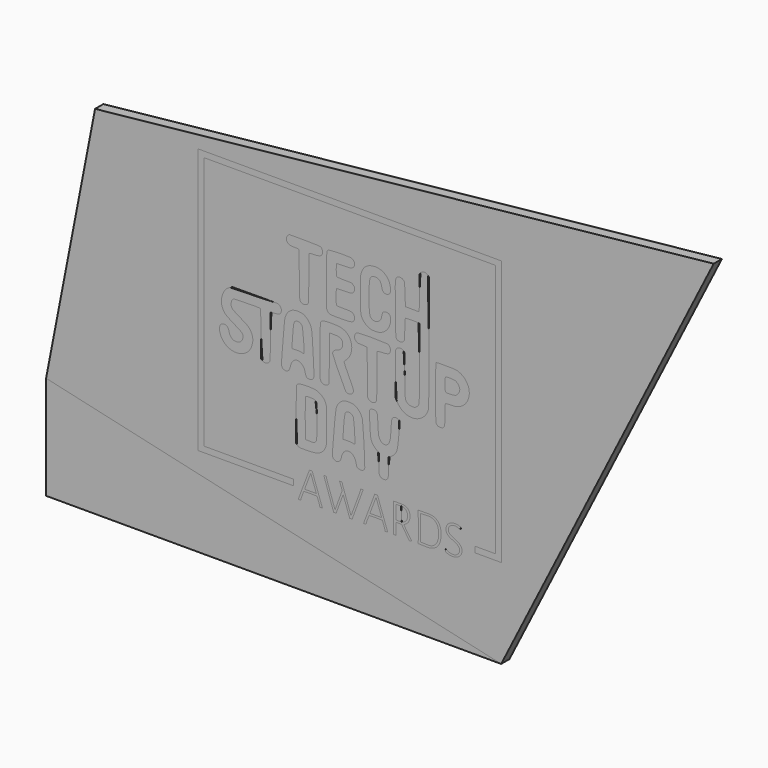
from build123d import *

# Parameters (mm, degrees)
F1_DEPTH = 6
F2_DEPTH = 6
F3_DEPTH = 6
F5_DEPTH = 6


# Not quite as in the source:
# - ends of sketch curves that miss each other by under 0.0002 mm in the source are joined


with BuildPart() as f1:
    # F0 (on Front) → F1 (new body)
    with BuildSketch(Plane.XZ):
        Polygon((70.674355, 83.849216), (-105.760285, 83.849216), (-105.760285, 82.155883), (-105.760285, -70.633826), (-50.198889, -70.633826), (-50.198889, -67.24716), (-102.373619, -67.24716), (-102.373619, 80.46255), (67.287688, 80.46255), (67.287688, -67.24716), (55.352222, -67.24716), (55.352222, -70.633826), (70.674355, -70.633826), align=None)
    extrude(amount=F1_DEPTH)


with BuildPart() as f1b:
    # F0 (on Front) → F1, piece 2 (new body)
    with BuildSketch(Plane.XZ):
        with BuildLine():
            add(Edge.make_bspline(
                [(-44.000473, 57.227722), (-34.335536, 57.227722), (-34.327284, 57.226593), (-33.601245, 55.696446)],
                knots=[0, 0, 0, 0, 1, 1, 1, 1], degree=3))
            Line((-44.000473, 57.227722), (-52.710226, 57.227722))
            Line((-52.710226, 57.227722), (-53.438938, 56.576737))
            add(Edge.make_bspline(
                [(-53.860618, 52.969584), (-54.643181, 53.961028), (-54.441996, 55.680509), (-53.438938, 56.576737)],
                knots=[0, 0, 0, 0, 1, 1, 1, 1], degree=3))
            add(Edge.make_bspline(
                [(-49.48507, 51.66541), (-52.095767, 51.66541), (-53.057162, 51.951662), (-53.860618, 52.969584)],
                knots=[0, 0, 0, 0, 1, 1, 1, 1], degree=3))
            add(Edge.make_bspline(
                [(-47.042637, 51.143959), (-47.158512, 51.641946), (-47.268923, 51.66541), (-49.48507, 51.66541)],
                knots=[0, 0, 0, 0, 1, 1, 1, 1], degree=3))
            add(Edge.make_bspline(
                [(-46.864594, 38.328206), (-46.895884, 45.089855), (-46.975891, 50.857151), (-47.042637, 51.143959)],
                knots=[0, 0, 0, 0, 1, 1, 1, 1], degree=3))
            add(Edge.make_bspline(
                [(-45.263313, 24.467897), (-46.868799, 25.278332), (-46.801509, 24.695992), (-46.864594, 38.328206)],
                knots=[0, 0, 0, 0, 1, 1, 1, 1], degree=3))
            add(Edge.make_bspline(
                [(-42.593226, 24.671294), (-43.445116, 24.113113), (-44.414691, 24.039515), (-45.263313, 24.467897)],
                knots=[0, 0, 0, 0, 1, 1, 1, 1], degree=3))
            add(Edge.make_bspline(
                [(-41.326533, 38.484198), (-41.347249, 25.098539), (-41.308838, 25.512864), (-42.593226, 24.671294)],
                knots=[0, 0, 0, 0, 1, 1, 1, 1], degree=3))
            add(Edge.make_bspline(
                [(-41.094471, 51.259715), (-41.215327, 51.02943), (-41.315668, 45.507744), (-41.326533, 38.484198)],
                knots=[0, 0, 0, 0, 1, 1, 1, 1], degree=3))
            add(Edge.make_bspline(
                [(-38.397928, 51.670371), (-40.524164, 51.666025), (-40.912214, 51.606984), (-41.094471, 51.259715)],
                knots=[0, 0, 0, 0, 1, 1, 1, 1], degree=3))
            add(Edge.make_bspline(
                [(-33.588573, 53.388509), (-34.12087, 52.114541), (-35.346705, 51.676637), (-38.397928, 51.670371)],
                knots=[0, 0, 0, 0, 1, 1, 1, 1], degree=3))
            add(Edge.make_bspline(
                [(-33.601245, 55.696446), (-33.163747, 54.7745), (-33.161579, 54.410441), (-33.588573, 53.388509)],
                knots=[0, 0, 0, 0, 1, 1, 1, 1], degree=3))
        make_face()
    extrude(amount=F1_DEPTH)


with BuildPart() as f1c:
    # F0 (on Front) → F1, piece 3 (new body)
    with BuildSketch(Plane.XZ):
        with BuildLine():
            add(Edge.make_bspline(
                [(-21.118976, 57.183074), (-18.967537, 57.199556), (-17.152363, 57.152275), (-16.734609, 57.014401)],
                knots=[0, 0, 0, 0, 1, 1, 1, 1], degree=3))
            add(Edge.make_bspline(
                [(-29.768721, 56.689733), (-29.224878, 56.950391), (-24.704782, 57.155589), (-21.118976, 57.183074)],
                knots=[0, 0, 0, 0, 1, 1, 1, 1], degree=3))
            add(Edge.make_bspline(
                [(-31.119749, 41.583678), (-31.041501, 56.164924), (-31.049535, 56.075854), (-29.768721, 56.689733)],
                knots=[0, 0, 0, 0, 1, 1, 1, 1], degree=3))
            add(Edge.make_bspline(
                [(-31.043132, 26.907019), (-31.125038, 27.585834), (-31.159421, 34.19043), (-31.119749, 41.583678)],
                knots=[0, 0, 0, 0, 1, 1, 1, 1], degree=3))
            add(Edge.make_bspline(
                [(-28.842679, 24.090862), (-30.04288, 24.373051), (-30.8642, 25.424241), (-31.043132, 26.907019)],
                knots=[0, 0, 0, 0, 1, 1, 1, 1], degree=3))
            add(Edge.make_bspline(
                [(-17.750575, 24.072123), (-19.89703, 23.823581), (-27.761895, 23.836758), (-28.842679, 24.090862)],
                knots=[0, 0, 0, 0, 1, 1, 1, 1], degree=3))
            add(Edge.make_bspline(
                [(-14.769603, 26.556451), (-14.929064, 24.879383), (-15.598831, 24.321291), (-17.750575, 24.072123)],
                knots=[0, 0, 0, 0, 1, 1, 1, 1], degree=3))
            add(Edge.make_bspline(
                [(-15.187975, 28.343491), (-14.758853, 27.799818), (-14.682475, 27.472748), (-14.769603, 26.556451)],
                knots=[0, 0, 0, 0, 1, 1, 1, 1], degree=3))
            add(Edge.make_bspline(
                [(-21.197874, 29.647665), (-16.847159, 29.647665), (-16.087584, 29.483229), (-15.187975, 28.343491)],
                knots=[0, 0, 0, 0, 1, 1, 1, 1], degree=3))
            add(Edge.make_bspline(
                [(-25.315454, 30.05336), (-25.169241, 29.689299), (-24.747685, 29.647665), (-21.197874, 29.647665)],
                knots=[0, 0, 0, 0, 1, 1, 1, 1], degree=3))
            add(Edge.make_bspline(
                [(-25.312632, 38.280801), (-25.52326, 37.747381), (-25.525611, 30.576809), (-25.315454, 30.05336)],
                knots=[0, 0, 0, 0, 1, 1, 1, 1], degree=3))
            add(Edge.make_bspline(
                [(-21.494916, 38.692007), (-24.759722, 38.687068), (-25.169709, 38.642835), (-25.312632, 38.280801)],
                knots=[0, 0, 0, 0, 1, 1, 1, 1], degree=3))
            add(Edge.make_bspline(
                [(-16.931956, 38.907532), (-17.430038, 38.791998), (-19.483267, 38.695055), (-21.494916, 38.692007)],
                knots=[0, 0, 0, 0, 1, 1, 1, 1], degree=3))
            add(Edge.make_bspline(
                [(-14.763476, 41.441467), (-14.899143, 40.029486), (-15.59359, 39.217968), (-16.931956, 38.907532)],
                knots=[0, 0, 0, 0, 1, 1, 1, 1], degree=3))
            add(Edge.make_bspline(
                [(-15.467378, 43.431907), (-14.701788, 42.66632), (-14.657781, 42.541402), (-14.763476, 41.441467)],
                knots=[0, 0, 0, 0, 1, 1, 1, 1], degree=3))
            add(Edge.make_bspline(
                [(-17.06094, 44.248807), (-16.481461, 44.248934), (-16.077099, 44.041631), (-15.467378, 43.431907)],
                knots=[0, 0, 0, 0, 1, 1, 1, 1], degree=3))
            add(Edge.make_bspline(
                [(-25.160497, 44.642375), (-24.919322, 44.401148), (-21.76463, 44.247961), (-17.06094, 44.248807)],
                knots=[0, 0, 0, 0, 1, 1, 1, 1], degree=3))
            add(Edge.make_bspline(
                [(-25.141193, 51.290032), (-25.469443, 50.960038), (-25.486851, 44.968807), (-25.160497, 44.642375)],
                knots=[0, 0, 0, 0, 1, 1, 1, 1], degree=3))
            add(Edge.make_bspline(
                [(-20.906206, 51.535322), (-23.12359, 51.51297), (-25.029422, 51.40239), (-25.141193, 51.290032)],
                knots=[0, 0, 0, 0, 1, 1, 1, 1], degree=3))
            add(Edge.make_bspline(
                [(-16.08197, 52.038581), (-16.783332, 51.628964), (-17.339835, 51.571269), (-20.906206, 51.535322)],
                knots=[0, 0, 0, 0, 1, 1, 1, 1], degree=3))
            add(Edge.make_bspline(
                [(-16.734609, 57.014401), (-14.356517, 56.229561), (-13.968831, 53.272716), (-16.08197, 52.038581)],
                knots=[0, 0, 0, 0, 1, 1, 1, 1], degree=3))
        make_face()
    extrude(amount=F1_DEPTH)


with BuildPart() as f1d:
    # F0 (on Front) → F1, piece 4 (new body)
    with BuildSketch(Plane.XZ):
        with BuildLine():
            add(Edge.make_bspline(
                [(-2.883119, 57.006685), (-0.898619, 57.042364), (1.097874, 56.521757), (2.561786, 55.415327)],
                knots=[0, 0, 0, 0, 1, 1, 1, 1], degree=3))
            add(Edge.make_bspline(
                [(-8.790493, 54.78694), (-7.365761, 56.211674), (-5.132218, 56.966249), (-2.883119, 57.006685)],
                knots=[0, 0, 0, 0, 1, 1, 1, 1], degree=3))
            add(Edge.make_bspline(
                [(-11.194343, 49.57961), (-10.934631, 51.473194), (-9.931695, 53.645735), (-8.790493, 54.78694)],
                knots=[0, 0, 0, 0, 1, 1, 1, 1], degree=3))
            add(Edge.make_bspline(
                [(-11.113864, 30.49764), (-11.339095, 32.093093), (-11.406391, 48.033732), (-11.194343, 49.57961)],
                knots=[0, 0, 0, 0, 1, 1, 1, 1], degree=3))
            add(Edge.make_bspline(
                [(-7.003453, 24.873038), (-8.996758, 25.89297), (-10.815121, 28.38147), (-11.113864, 30.49764)],
                knots=[0, 0, 0, 0, 1, 1, 1, 1], degree=3))
            add(Edge.make_bspline(
                [(-2.193548, 23.949204), (-4.40216, 23.861246), (-5.401111, 24.053163), (-7.003453, 24.873038)],
                knots=[0, 0, 0, 0, 1, 1, 1, 1], degree=3))
            add(Edge.make_bspline(
                [(1.16721, 24.68783), (0.052639, 24.158926), (-0.614568, 24.012083), (-2.193548, 23.949204)],
                knots=[0, 0, 0, 0, 1, 1, 1, 1], degree=3))
            add(Edge.make_bspline(
                [(6.185474, 31.526207), (5.680765, 28.479658), (3.822868, 25.948031), (1.16721, 24.68783)],
                knots=[0, 0, 0, 0, 1, 1, 1, 1], degree=3))
            add(Edge.make_bspline(
                [(3.376483, 35.825134), (5.614852, 36.053847), (6.668402, 34.441269), (6.185474, 31.526207)],
                knots=[0, 0, 0, 0, 1, 1, 1, 1], degree=3))
            add(Edge.make_bspline(
                [(1.04925, 32.87889), (1.405539, 34.991283), (1.948565, 35.679237), (3.376483, 35.825134)],
                knots=[0, 0, 0, 0, 1, 1, 1, 1], degree=3))
            add(Edge.make_bspline(
                [(-0.00853, 30.354875), (0.618686, 31.049119), (0.822676, 31.535661), (1.04925, 32.87889)],
                knots=[0, 0, 0, 0, 1, 1, 1, 1], degree=3))
            add(Edge.make_bspline(
                [(-5.571949, 30.609538), (-4.553234, 28.639582), (-1.677135, 28.507933), (-0.00853, 30.354875)],
                knots=[0, 0, 0, 0, 1, 1, 1, 1], degree=3))
            add(Edge.make_bspline(
                [(-6.355225, 40.540783), (-6.352968, 35.143887), (-6.071631, 31.575819), (-5.571949, 30.609538)],
                knots=[0, 0, 0, 0, 1, 1, 1, 1], degree=3))
            add(Edge.make_bspline(
                [(-5.549899, 50.282411), (-6.076373, 49.264308), (-6.357483, 45.866296), (-6.355225, 40.540783)],
                knots=[0, 0, 0, 0, 1, 1, 1, 1], degree=3))
            add(Edge.make_bspline(
                [(-2.786105, 51.764628), (-4.157493, 51.764628), (-5.023588, 51.300175), (-5.549899, 50.282411)],
                knots=[0, 0, 0, 0, 1, 1, 1, 1], degree=3))
            add(Edge.make_bspline(
                [(1.07185, 47.91935), (0.650064, 50.576331), (-0.54215, 51.764628), (-2.786105, 51.764628)],
                knots=[0, 0, 0, 0, 1, 1, 1, 1], degree=3))
            add(Edge.make_bspline(
                [(3.740284, 45.060196), (2.207911, 45.060196), (1.385981, 45.940676), (1.07185, 47.91935)],
                knots=[0, 0, 0, 0, 1, 1, 1, 1], degree=3))
            add(Edge.make_bspline(
                [(5.473857, 45.817015), (4.897299, 45.171739), (4.64182, 45.060196), (3.740284, 45.060196)],
                knots=[0, 0, 0, 0, 1, 1, 1, 1], degree=3))
            add(Edge.make_bspline(
                [(6.150197, 48.29969), (6.150197, 46.720267), (6.092759, 46.509673), (5.473857, 45.817015)],
                knots=[0, 0, 0, 0, 1, 1, 1, 1], degree=3))
            add(Edge.make_bspline(
                [(2.561786, 55.415327), (4.946423, 53.613023), (6.150197, 51.226506), (6.150197, 48.29969)],
                knots=[0, 0, 0, 0, 1, 1, 1, 1], degree=3))
        make_face()
    extrude(amount=F1_DEPTH)


with BuildPart() as f1e:
    # F0 (on Front) → F1, piece 5 (new body)
    with BuildSketch(Plane.XZ):
        with BuildLine():
            add(Edge.make_bspline(
                [(25.612506, 63.484016), (26.385394, 63.5197), (27.199797, 63.205434), (27.84548, 62.531516)],
                knots=[0, 0, 0, 0, 1, 1, 1, 1], degree=3))
            add(Edge.make_bspline(
                [(23.627615, 62.336923), (24.108002, 63.062827), (24.839649, 63.448317), (25.612506, 63.484016)],
                knots=[0, 0, 0, 0, 1, 1, 1, 1], degree=3))
            Line((23.627615, 62.336923), (23.032292, 52.213302))
            add(Edge.make_bspline(
                [(22.805744, 42.567587), (22.936966, 42.812765), (23.030035, 46.769173), (23.032292, 52.213302)],
                knots=[0, 0, 0, 0, 1, 1, 1, 1], degree=3))
            add(Edge.make_bspline(
                [(18.712419, 42.21536), (22.235542, 42.157572), (22.603275, 42.189282), (22.805744, 42.567587)],
                knots=[0, 0, 0, 0, 1, 1, 1, 1], degree=3))
            Line((18.712419, 42.21536), (14.841233, 42.278749))
            Line((14.841233, 42.278749), (14.658229, 48.188881))
            add(Edge.make_bspline(
                [(14.213398, 54.763775), (14.363625, 54.382693), (14.553313, 51.57684), (14.658229, 48.188881)],
                knots=[0, 0, 0, 0, 1, 1, 1, 1], degree=3))
            add(Edge.make_bspline(
                [(11.758838, 56.299462), (12.761676, 56.298333), (13.885544, 55.595501), (14.213398, 54.763775)],
                knots=[0, 0, 0, 0, 1, 1, 1, 1], degree=3))
            add(Edge.make_bspline(
                [(9.262382, 54.551008), (9.716244, 55.739417), (10.518046, 56.300873), (11.758838, 56.299462)],
                knots=[0, 0, 0, 0, 1, 1, 1, 1], degree=3))
            add(Edge.make_bspline(
                [(9.01103, 39.191944), (8.866806, 52.48128), (8.88456, 53.561706), (9.262382, 54.551008)],
                knots=[0, 0, 0, 0, 1, 1, 1, 1], degree=3))
            add(Edge.make_bspline(
                [(10.901698, 23.44207), (9.077118, 24.052714), (9.185107, 23.155454), (9.01103, 39.191944)],
                knots=[0, 0, 0, 0, 1, 1, 1, 1], degree=3))
            add(Edge.make_bspline(
                [(13.822035, 24.225897), (13.004073, 23.356074), (11.979768, 23.081266), (10.901698, 23.44207)],
                knots=[0, 0, 0, 0, 1, 1, 1, 1], degree=3))
            add(Edge.make_bspline(
                [(14.493417, 30.486052), (14.379179, 24.897913), (14.369668, 24.808243), (13.822035, 24.225897)],
                knots=[0, 0, 0, 0, 1, 1, 1, 1], degree=3))
            add(Edge.make_bspline(
                [(14.956989, 36.374133), (14.66884, 36.192345), (14.58946, 35.184798), (14.493417, 30.486052)],
                knots=[0, 0, 0, 0, 1, 1, 1, 1], degree=3))
            add(Edge.make_bspline(
                [(22.474463, 36.374697), (21.712379, 36.664271), (15.416368, 36.663958), (14.956989, 36.374133)],
                knots=[0, 0, 0, 0, 1, 1, 1, 1], degree=3))
            Line((22.474463, 36.374697), (23.068674, 36.148699))
            Line((23.068674, 36.148699), (23.066416, 16.037609))
            add(Edge.make_bspline(
                [(22.830498, -4.920146), (22.981049, -4.37811), (23.066416, 3.156738), (23.066416, 16.037609)],
                knots=[0, 0, 0, 0, 1, 1, 1, 1], degree=3))
            add(Edge.make_bspline(
                [(20.165922, -7.572044), (21.091145, -7.339832), (22.566078, -5.872135), (22.830498, -4.920146)],
                knots=[0, 0, 0, 0, 1, 1, 1, 1], degree=3))
            add(Edge.make_bspline(
                [(16.247332, -6.883024), (17.118365, -7.547381), (18.968078, -7.872684), (20.165922, -7.572044)],
                knots=[0, 0, 0, 0, 1, 1, 1, 1], degree=3))
            add(Edge.make_bspline(
                [(14.492815, 6.858774), (14.621859, -6.090273), (14.558426, -5.594838), (16.247332, -6.883024)],
                knots=[0, 0, 0, 0, 1, 1, 1, 1], degree=3))
            Line((14.492815, 6.858774), (13.811511, 19.088036))
            add(Edge.make_bspline(
                [(12.385519, 19.94793), (12.858709, 19.806159), (13.500468, 19.418947), (13.811511, 19.088036)],
                knots=[0, 0, 0, 0, 1, 1, 1, 1], degree=3))
            add(Edge.make_bspline(
                [(10.633206, 19.769888), (11.382357, 20.135743), (11.662719, 20.164482), (12.385519, 19.94793)],
                knots=[0, 0, 0, 0, 1, 1, 1, 1], degree=3))
            add(Edge.make_bspline(
                [(8.983417, 5.89194), (8.912356, 19.232186), (8.873892, 18.910724), (10.633206, 19.769888)],
                knots=[0, 0, 0, 0, 1, 1, 1, 1], degree=3))
            Line((8.983417, 5.89194), (9.831738, -7.603461))
            add(Edge.make_bspline(
                [(20.513739, -13.229166), (16.179649, -14.05111), (11.763763, -11.725401), (9.831738, -7.603461)],
                knots=[0, 0, 0, 0, 1, 1, 1, 1], degree=3))
            Line((20.513739, -13.229166), (20.514867, -13.229166))
            add(Edge.make_bspline(
                [(28.403309, -5.31647), (27.662038, -9.326394), (24.530675, -12.467584), (20.514867, -13.229166)],
                knots=[0, 0, 0, 0, 1, 1, 1, 1], degree=3))
            add(Edge.make_bspline(
                [(28.57584, 28.886439), (28.614846, 7.584791), (28.553601, -4.503495), (28.403309, -5.31647)],
                knots=[0, 0, 0, 0, 1, 1, 1, 1], degree=3))
            Line((28.57584, 28.886439), (27.84548, 62.531516))
        make_face()
    extrude(amount=F1_DEPTH)


with BuildPart() as f1f:
    # F0 (on Front) → F1, piece 6 (new body)
    with BuildSketch(Plane.XZ):
        with BuildLine():
            add(Edge.make_bspline(
                [(-58.503498, 19.162449), (-57.44403, 18.44948), (-57.020598, 17.237104), (-57.417052, 16.053594)],
                knots=[0, 0, 0, 0, 1, 1, 1, 1], degree=3))
            Line((-58.503498, 19.162449), (-59.306618, 19.70319))
            Line((-59.306618, 19.70319), (-87.046519, 18.955191))
            add(Edge.make_bspline(
                [(-92.218572, 11.094312), (-91.680896, 14.99994), (-89.98524, 17.577258), (-87.046519, 18.955191)],
                knots=[0, 0, 0, 0, 1, 1, 1, 1], degree=3))
            add(Edge.make_bspline(
                [(-90.334518, 4.927866), (-91.712914, 6.738412), (-92.474841, 9.232782), (-92.218572, 11.094312)],
                knots=[0, 0, 0, 0, 1, 1, 1, 1], degree=3))
            add(Edge.make_bspline(
                [(-83.626229, 0.255214), (-87.40828, 2.474686), (-89.661799, 4.04424), (-90.334518, 4.927866)],
                knots=[0, 0, 0, 0, 1, 1, 1, 1], degree=3))
            add(Edge.make_bspline(
                [(-79.602358, -3.751571), (-79.602358, -2.419457), (-80.368111, -1.65679), (-83.626229, 0.255214)],
                knots=[0, 0, 0, 0, 1, 1, 1, 1], degree=3))
            add(Edge.make_bspline(
                [(-83.210061, -7.618896), (-81.036315, -7.438632), (-79.602358, -5.90161), (-79.602358, -3.751571)],
                knots=[0, 0, 0, 0, 1, 1, 1, 1], degree=3))
            add(Edge.make_bspline(
                [(-85.160812, -7.435894), (-84.763248, -7.600571), (-83.930083, -7.678606), (-83.210061, -7.618896)],
                knots=[0, 0, 0, 0, 1, 1, 1, 1], degree=3))
            add(Edge.make_bspline(
                [(-87.604348, -4.492954), (-87.431778, -5.519058), (-86.196593, -7.00686), (-85.160812, -7.435894)],
                knots=[0, 0, 0, 0, 1, 1, 1, 1], degree=3))
            add(Edge.make_bspline(
                [(-90.597448, -0.944783), (-88.902853, -0.944783), (-88.026353, -1.983742), (-87.604348, -4.492954)],
                knots=[0, 0, 0, 0, 1, 1, 1, 1], degree=3))
            add(Edge.make_bspline(
                [(-92.389999, -7.767173), (-94.099521, -4.114009), (-93.26683, -0.944783), (-90.597448, -0.944783)],
                knots=[0, 0, 0, 0, 1, 1, 1, 1], degree=3))
            add(Edge.make_bspline(
                [(-80.065928, -12.666375), (-84.920748, -14.424727), (-90.269669, -12.298214), (-92.389999, -7.767173)],
                knots=[0, 0, 0, 0, 1, 1, 1, 1], degree=3))
            add(Edge.make_bspline(
                [(-74.040043, -5.131262), (-74.69801, -8.796917), (-76.865378, -11.507176), (-80.065928, -12.666375)],
                knots=[0, 0, 0, 0, 1, 1, 1, 1], degree=3))
            add(Edge.make_bspline(
                [(-77.32308, 2.954515), (-74.745127, 1.013808), (-73.491394, -2.074649), (-74.040043, -5.131262)],
                knots=[0, 0, 0, 0, 1, 1, 1, 1], degree=3))
            add(Edge.make_bspline(
                [(-81.431288, 5.531997), (-79.851806, 4.625942), (-78.00294, 3.466316), (-77.32308, 2.954515)],
                knots=[0, 0, 0, 0, 1, 1, 1, 1], degree=3))
            add(Edge.make_bspline(
                [(-86.500817, 11.126832), (-86.716892, 8.878097), (-86.125323, 8.22469), (-81.431288, 5.531997)],
                knots=[0, 0, 0, 0, 1, 1, 1, 1], degree=3))
            add(Edge.make_bspline(
                [(-84.67905, 13.816763), (-85.751139, 13.441111), (-86.365576, 12.534263), (-86.500817, 11.126832)],
                knots=[0, 0, 0, 0, 1, 1, 1, 1], degree=3))
            add(Edge.make_bspline(
                [(-69.636386, 13.89283), (-70.165106, 14.226905), (-83.703936, 14.158438), (-84.67905, 13.816763)],
                knots=[0, 0, 0, 0, 1, 1, 1, 1], degree=3))
            add(Edge.make_bspline(
                [(-69.172813, 1.014237), (-69.272723, 11.928527), (-69.336652, 13.703442), (-69.636386, 13.89283)],
                knots=[0, 0, 0, 0, 1, 1, 1, 1], degree=3))
            Line((-69.172813, 1.014237), (-68.300238, -12.320763))
            add(Edge.make_bspline(
                [(-63.835395, -10.794999), (-64.324185, -12.913139), (-66.720195, -13.731866), (-68.300238, -12.320763)],
                knots=[0, 0, 0, 0, 1, 1, 1, 1], degree=3))
            add(Edge.make_bspline(
                [(-63.61601, 2.005322), (-63.619058, -4.525077), (-63.717734, -10.28512), (-63.835395, -10.794999)],
                knots=[0, 0, 0, 0, 1, 1, 1, 1], degree=3))
            Line((-63.61601, 2.005322), (-63.610507, 13.879052))
            Line((-63.610507, 13.879052), (-63.089059, 13.989844))
            add(Edge.make_bspline(
                [(-60.783326, 14.172298), (-61.764751, 14.133108), (-62.802253, 14.050835), (-63.089059, 13.989844)],
                knots=[0, 0, 0, 0, 1, 1, 1, 1], degree=3))
            add(Edge.make_bspline(
                [(-57.417052, 16.053594), (-57.86429, 14.718491), (-58.692773, 14.255779), (-60.783326, 14.172298)],
                knots=[0, 0, 0, 0, 1, 1, 1, 1], degree=3))
        make_face()
    extrude(amount=F1_DEPTH)


with BuildPart() as f1g:
    # F0 (on Front) → F1, piece 7 (new body)
    with BuildSketch(Plane.XZ):
        with BuildLine():
            add(Edge.make_bspline(
                [(-47.754249, 19.587428), (-46.54936, 19.592734), (-45.348717, 19.41527), (-44.555548, 19.05385)],
                knots=[0, 0, 0, 0, 1, 1, 1, 1], degree=3))
            add(Edge.make_bspline(
                [(-50.979408, 19.025732), (-50.168293, 19.39421), (-48.959135, 19.582119), (-47.754249, 19.587428)],
                knots=[0, 0, 0, 0, 1, 1, 1, 1], degree=3))
            add(Edge.make_bspline(
                [(-55.125651, 13.887857), (-54.428683, 16.367202), (-53.037551, 18.090753), (-50.979408, 19.025732)],
                knots=[0, 0, 0, 0, 1, 1, 1, 1], degree=3))
            add(Edge.make_bspline(
                [(-56.895602, -5.059617), (-55.667977, 10.464174), (-55.459192, 12.701355), (-55.125651, 13.887857)],
                knots=[0, 0, 0, 0, 1, 1, 1, 1], degree=3))
            add(Edge.make_bspline(
                [(-55.913339, -12.879157), (-57.355438, -12.252592), (-57.42224, -11.719164), (-56.895602, -5.059617)],
                knots=[0, 0, 0, 0, 1, 1, 1, 1], degree=3))
            add(Edge.make_bspline(
                [(-53.76856, -12.898997), (-54.731632, -13.301398), (-54.946186, -13.29936), (-55.913339, -12.879157)],
                knots=[0, 0, 0, 0, 1, 1, 1, 1], degree=3))
            add(Edge.make_bspline(
                [(-51.999709, -9.937317), (-52.362128, -11.684403), (-52.860789, -12.519704), (-53.76856, -12.898997)],
                knots=[0, 0, 0, 0, 1, 1, 1, 1], degree=3))
            add(Edge.make_bspline(
                [(-45.036206, -7.197775), (-47.759541, -4.386757), (-51.122769, -5.709916), (-51.999709, -9.937317)],
                knots=[0, 0, 0, 0, 1, 1, 1, 1], degree=3))
            add(Edge.make_bspline(
                [(-43.573832, -10.015589), (-43.907323, -8.541884), (-44.10671, -8.157204), (-45.036206, -7.197775)],
                knots=[0, 0, 0, 0, 1, 1, 1, 1], degree=3))
            add(Edge.make_bspline(
                [(-42.85615, -12.232027), (-43.03846, -11.951543), (-43.36144, -10.954173), (-43.573832, -10.015589)],
                knots=[0, 0, 0, 0, 1, 1, 1, 1], degree=3))
            add(Edge.make_bspline(
                [(-38.822356, -12.146037), (-39.750785, -13.326346), (-42.112062, -13.37681), (-42.85615, -12.232027)],
                knots=[0, 0, 0, 0, 1, 1, 1, 1], degree=3))
            add(Edge.make_bspline(
                [(-38.812986, 0.615149), (-38.20819, -10.179998), (-38.208805, -11.366034), (-38.822356, -12.146037)],
                knots=[0, 0, 0, 0, 1, 1, 1, 1], degree=3))
            add(Edge.make_bspline(
                [(-40.410409, 14.881152), (-39.559052, 13.097296), (-39.465094, 12.254555), (-38.812986, 0.615149)],
                knots=[0, 0, 0, 0, 1, 1, 1, 1], degree=3))
            add(Edge.make_bspline(
                [(-44.555548, 19.05385), (-42.930944, 18.313581), (-41.232726, 16.604164), (-40.410409, 14.881152)],
                knots=[0, 0, 0, 0, 1, 1, 1, 1], degree=3))
        make_face()
        with BuildLine():
            add(Edge.make_bspline(
                [(-47.881029, 14.387814), (-48.672236, 14.366111), (-49.412319, 13.981978), (-49.813588, 13.206008)],
                knots=[0, 0, 0, 0, 1, 1, 1, 1], degree=3))
            add(Edge.make_bspline(
                [(-45.188894, 12.736374), (-45.762025, 13.844688), (-46.863762, 14.415728), (-47.881029, 14.387814)],
                knots=[0, 0, 0, 0, 1, 1, 1, 1], degree=3))
            add(Edge.make_bspline(
                [(-44.255134, -0.826278), (-43.819662, -0.300662), (-44.64475, 11.684116), (-45.188894, 12.736374)],
                knots=[0, 0, 0, 0, 1, 1, 1, 1], degree=3))
            add(Edge.make_bspline(
                [(-45.532852, -0.778323), (-44.713731, -1.038667), (-44.439761, -1.049127), (-44.255134, -0.826278)],
                knots=[0, 0, 0, 0, 1, 1, 1, 1], degree=3))
            add(Edge.make_bspline(
                [(-48.835733, -0.570514), (-47.219012, -0.482136), (-46.279031, -0.541155), (-45.532852, -0.778323)],
                knots=[0, 0, 0, 0, 1, 1, 1, 1], degree=3))
            add(Edge.make_bspline(
                [(-51.147531, 0.445376), (-51.216162, -0.711738), (-51.238872, -0.701875), (-48.835733, -0.570514)],
                knots=[0, 0, 0, 0, 1, 1, 1, 1], degree=3))
            add(Edge.make_bspline(
                [(-49.813588, 13.206008), (-50.255517, 12.351414), (-50.685214, 8.239927), (-51.147531, 0.445376)],
                knots=[0, 0, 0, 0, 1, 1, 1, 1], degree=3))
        make_face(mode=Mode.SUBTRACT)
    extrude(amount=F1_DEPTH)


with BuildPart() as f1h:
    # F0 (on Front) → F1, piece 8 (new body)
    with BuildSketch(Plane.XZ):
        with BuildLine():
            add(Edge.make_bspline(
                [(-28.155239, 19.765479), (-23.874512, 19.799741), (-22.588285, 19.587095), (-20.44098, 18.491621)],
                knots=[0, 0, 0, 0, 1, 1, 1, 1], degree=3))
            add(Edge.make_bspline(
                [(-34.332708, 18.379181), (-33.58605, 19.518312), (-32.64472, 19.729561), (-28.155239, 19.765479)],
                knots=[0, 0, 0, 0, 1, 1, 1, 1], degree=3))
            add(Edge.make_bspline(
                [(-34.827148, 4.280197), (-34.760549, 16.85077), (-34.728545, 17.775279), (-34.332708, 18.379181)],
                knots=[0, 0, 0, 0, 1, 1, 1, 1], degree=3))
            add(Edge.make_bspline(
                [(-34.752734, -10.388193), (-34.832888, -9.719702), (-34.866348, -3.118786), (-34.827148, 4.280197)],
                knots=[0, 0, 0, 0, 1, 1, 1, 1], degree=3))
            add(Edge.make_bspline(
                [(-32.12454, -12.996544), (-33.644749, -12.996544), (-34.547398, -12.100799), (-34.752734, -10.388193)],
                knots=[0, 0, 0, 0, 1, 1, 1, 1], degree=3))
            add(Edge.make_bspline(
                [(-29.716831, -11.767884), (-30.194924, -12.603663), (-30.964925, -12.996544), (-32.12454, -12.996544)],
                knots=[0, 0, 0, 0, 1, 1, 1, 1], degree=3))
            add(Edge.make_bspline(
                [(-29.309483, 1.604598), (-29.397136, -8.124979), (-29.496337, -11.382434), (-29.716831, -11.767884)],
                knots=[0, 0, 0, 0, 1, 1, 1, 1], degree=3))
            Line((-29.309483, 1.604598), (-29.193727, 14.467206))
            Line((-29.193727, 14.467206), (-26.644357, 14.45507))
            add(Edge.make_bspline(
                [(-21.661371, 11.211168), (-21.661371, 13.68271), (-22.819038, 14.436472), (-26.644357, 14.45507)],
                knots=[0, 0, 0, 0, 1, 1, 1, 1], degree=3))
            add(Edge.make_bspline(
                [(-24.998979, 7.067683), (-22.803205, 7.706008), (-21.661371, 9.12354), (-21.661371, 11.211168)],
                knots=[0, 0, 0, 0, 1, 1, 1, 1], degree=3))
            add(Edge.make_bspline(
                [(-27.455746, 4.591624), (-27.455746, 5.646793), (-26.469901, 6.640074), (-24.998979, 7.067683)],
                knots=[0, 0, 0, 0, 1, 1, 1, 1], degree=3))
            add(Edge.make_bspline(
                [(-20.069463, -12.030272), (-21.994895, -8.546461), (-27.455746, 3.742355), (-27.455746, 4.591624)],
                knots=[0, 0, 0, 0, 1, 1, 1, 1], degree=3))
            add(Edge.make_bspline(
                [(-16.041181, -12.305879), (-17.131004, -13.514792), (-19.332329, -13.364015), (-20.069463, -12.030272)],
                knots=[0, 0, 0, 0, 1, 1, 1, 1], degree=3))
            add(Edge.make_bspline(
                [(-16.298598, -7.872456), (-15.198282, -10.263549), (-15.137892, -11.303883), (-16.041181, -12.305879)],
                knots=[0, 0, 0, 0, 1, 1, 1, 1], degree=3))
            add(Edge.make_bspline(
                [(-19.087197, -1.804127), (-18.045644, -4.072336), (-16.790732, -6.803003), (-16.298598, -7.872456)],
                knots=[0, 0, 0, 0, 1, 1, 1, 1], degree=3))
            add(Edge.make_bspline(
                [(-20.809743, 2.599533), (-20.906505, 2.441279), (-20.159525, 0.531109), (-19.087197, -1.804127)],
                knots=[0, 0, 0, 0, 1, 1, 1, 1], degree=3))
            add(Edge.make_bspline(
                [(-19.397531, 4.016706), (-20.080483, 3.391053), (-20.715754, 2.753248), (-20.809743, 2.599533)],
                knots=[0, 0, 0, 0, 1, 1, 1, 1], degree=3))
            add(Edge.make_bspline(
                [(-20.44098, 18.491621), (-15.480972, 15.961211), (-14.916057, 8.122173), (-19.397531, 4.016706)],
                knots=[0, 0, 0, 0, 1, 1, 1, 1], degree=3))
        make_face()
    extrude(amount=F1_DEPTH)


with BuildPart() as f1i:
    # F0 (on Front) → F1, piece 9 (new body)
    with BuildSketch(Plane.XZ):
        with BuildLine():
            add(Edge.make_bspline(
                [(-4.306357, 20.062583), (0.026528, 20.07009), (4.358752, 19.958816), (4.801372, 19.721932)],
                knots=[0, 0, 0, 0, 1, 1, 1, 1], degree=3))
            add(Edge.make_bspline(
                [(-13.418497, 19.689962), (-12.973001, 19.928384), (-8.639241, 20.055073), (-4.306357, 20.062583)],
                knots=[0, 0, 0, 0, 1, 1, 1, 1], degree=3))
            add(Edge.make_bspline(
                [(-14.708341, 17.120747), (-14.708341, 18.32097), (-14.242559, 19.248936), (-13.418497, 19.689962)],
                knots=[0, 0, 0, 0, 1, 1, 1, 1], degree=3))
            add(Edge.make_bspline(
                [(-13.920656, 15.371189), (-14.563617, 16.014148), (-14.708341, 16.336022), (-14.708341, 17.120747)],
                knots=[0, 0, 0, 0, 1, 1, 1, 1], degree=3))
            add(Edge.make_bspline(
                [(-9.677949, 14.456174), (-13.173429, 14.55531), (-13.085827, 14.536361), (-13.920656, 15.371189)],
                knots=[0, 0, 0, 0, 1, 1, 1, 1], degree=3))
            add(Edge.make_bspline(
                [(-7.65003, 14.271516), (-7.84675, 14.347004), (-8.75931, 14.430125), (-9.677949, 14.456174)],
                knots=[0, 0, 0, 0, 1, 1, 1, 1], degree=3))
            add(Edge.make_bspline(
                [(-7.292291, 1.59632), (-7.292291, 12.683516), (-7.333718, 14.15014), (-7.65003, 14.271516)],
                knots=[0, 0, 0, 0, 1, 1, 1, 1], degree=3))
            add(Edge.make_bspline(
                [(-7.038731, -11.447638), (-7.212995, -11.099788), (-7.292291, -7.018826), (-7.292291, 1.59632)],
                knots=[0, 0, 0, 0, 1, 1, 1, 1], degree=3))
            add(Edge.make_bspline(
                [(-6.169464, -12.474001), (-6.508001, -12.187828), (-6.899257, -11.726064), (-7.038731, -11.447638)],
                knots=[0, 0, 0, 0, 1, 1, 1, 1], degree=3))
            add(Edge.make_bspline(
                [(-2.938793, -12.634956), (-3.725306, -13.185856), (-5.427727, -13.101023), (-6.169464, -12.474001)],
                knots=[0, 0, 0, 0, 1, 1, 1, 1], degree=3))
            add(Edge.make_bspline(
                [(-1.726118, 1.418828), (-1.729956, -11.883652), (-1.721263, -11.782167), (-2.938793, -12.634956)],
                knots=[0, 0, 0, 0, 1, 1, 1, 1], degree=3))
            add(Edge.make_bspline(
                [(-1.552486, 14.03284), (-1.646141, 13.889336), (-1.72386, 8.212921), (-1.726118, 1.418828)],
                knots=[0, 0, 0, 0, 1, 1, 1, 1], degree=3))
            add(Edge.make_bspline(
                [(1.399273, 14.396091), (-0.29772, 14.33363), (-1.448589, 14.192045), (-1.552486, 14.03284)],
                knots=[0, 0, 0, 0, 1, 1, 1, 1], degree=3))
            add(Edge.make_bspline(
                [(5.873486, 15.8513), (5.401153, 14.814641), (4.460795, 14.508774), (1.399273, 14.396091)],
                knots=[0, 0, 0, 0, 1, 1, 1, 1], degree=3))
            add(Edge.make_bspline(
                [(4.801372, 19.721932), (5.997596, 19.081731), (6.507126, 17.241989), (5.873486, 15.8513)],
                knots=[0, 0, 0, 0, 1, 1, 1, 1], degree=3))
        make_face()
    extrude(amount=F1_DEPTH)


with BuildPart() as f1j:
    # F0 (on Front) → F1, piece 10 (new body)
    with BuildSketch(Plane.XZ):
        with BuildLine():
            add(Edge.make_bspline(
                [(38.271164, 19.681685), (42.970371, 19.681685), (43.833751, 19.624526), (45.129936, 19.224177)],
                knots=[0, 0, 0, 0, 1, 1, 1, 1], degree=3))
            add(Edge.make_bspline(
                [(32.617349, 19.403874), (32.817685, 19.604198), (34.399094, 19.681685), (38.271164, 19.681685)],
                knots=[0, 0, 0, 0, 1, 1, 1, 1], degree=3))
            add(Edge.make_bspline(
                [(32.339538, 4.331993), (32.339538, 15.529372), (32.40684, 19.19337), (32.617349, 19.403874)],
                knots=[0, 0, 0, 0, 1, 1, 1, 1], degree=3))
            add(Edge.make_bspline(
                [(33.565441, -12.585905), (32.339598, -11.627075), (32.339538, -11.641703), (32.339538, 4.331993)],
                knots=[0, 0, 0, 0, 1, 1, 1, 1], degree=3))
            add(Edge.make_bspline(
                [(36.661066, -12.657014), (35.992964, -13.124975), (34.202603, -13.083853), (33.565441, -12.585905)],
                knots=[0, 0, 0, 0, 1, 1, 1, 1], degree=3))
            add(Edge.make_bspline(
                [(37.90185, -5.379319), (37.90185, -11.101239), (37.768757, -11.881163), (36.661066, -12.657014)],
                knots=[0, 0, 0, 0, 1, 1, 1, 1], degree=3))
            add(Edge.make_bspline(
                [(38.349988, 0.205597), (37.926638, -0.020954), (37.90185, -0.331763), (37.90185, -5.379319)],
                knots=[0, 0, 0, 0, 1, 1, 1, 1], degree=3))
            add(Edge.make_bspline(
                [(41.305052, 0.44813), (39.926363, 0.446719), (38.596538, 0.337553), (38.349988, 0.205597)],
                knots=[0, 0, 0, 0, 1, 1, 1, 1], degree=3))
            add(Edge.make_bspline(
                [(49.476268, 3.603287), (47.416819, 1.34992), (45.090741, 0.451912), (41.305052, 0.44813)],
                knots=[0, 0, 0, 0, 1, 1, 1, 1], degree=3))
            add(Edge.make_bspline(
                [(45.129936, 19.224177), (51.984936, 17.106884), (54.279721, 8.859041), (49.476268, 3.603287)],
                knots=[0, 0, 0, 0, 1, 1, 1, 1], degree=3))
        make_face()
        with BuildLine():
            add(Edge.make_bspline(
                [(39.947962, 14.107796), (38.952076, 14.107231), (38.427726, 14.03562), (38.246359, 13.885105)],
                knots=[0, 0, 0, 0, 1, 1, 1, 1], degree=3))
            add(Edge.make_bspline(
                [(41.106066, 14.085195), (40.664671, 14.100294), (40.279923, 14.108027), (39.947962, 14.107796)],
                knots=[0, 0, 0, 0, 1, 1, 1, 1], degree=3))
            add(Edge.make_bspline(
                [(44.557222, 13.379089), (43.715712, 13.935984), (43.366496, 14.007827), (41.106066, 14.085195)],
                knots=[0, 0, 0, 0, 1, 1, 1, 1], degree=3))
            add(Edge.make_bspline(
                [(46.477107, 10.098806), (46.477107, 11.15747), (45.568289, 12.71), (44.557222, 13.379089)],
                knots=[0, 0, 0, 0, 1, 1, 1, 1], degree=3))
            add(Edge.make_bspline(
                [(43.831273, 6.254632), (45.157469, 6.677034), (46.477107, 8.59393), (46.477107, 10.098806)],
                knots=[0, 0, 0, 0, 1, 1, 1, 1], degree=3))
            add(Edge.make_bspline(
                [(38.712689, 5.943747), (39.393494, 5.770994), (43.001074, 5.990215), (43.831273, 6.254632)],
                knots=[0, 0, 0, 0, 1, 1, 1, 1], degree=3))
            add(Edge.make_bspline(
                [(38.079343, 6.324637), (38.172998, 6.180047), (38.457749, 6.008438), (38.712689, 5.943747)],
                knots=[0, 0, 0, 0, 1, 1, 1, 1], degree=3))
            add(Edge.make_bspline(
                [(37.905158, 10.093295), (37.907134, 8.164986), (37.985687, 6.469228), (38.079343, 6.324637)],
                knots=[0, 0, 0, 0, 1, 1, 1, 1], degree=3))
            add(Edge.make_bspline(
                [(38.246359, 13.885105), (37.969056, 13.65495), (37.902336, 12.915816), (37.905158, 10.093295)],
                knots=[0, 0, 0, 0, 1, 1, 1, 1], degree=3))
        make_face(mode=Mode.SUBTRACT)
    extrude(amount=F1_DEPTH)


with BuildPart() as f1k:
    # F0 (on Front) → F1, piece 11 (new body)
    with BuildSketch(Plane.XZ):
        with BuildLine():
            add(Edge.make_bspline(
                [(9.311416, -16.401409), (9.944971, -16.413657), (10.576262, -16.622803), (10.978291, -17.024835)],
                knots=[0, 0, 0, 0, 1, 1, 1, 1], degree=3))
            add(Edge.make_bspline(
                [(7.63076, -16.960341), (8.041966, -16.57403), (8.677863, -16.389163), (9.311416, -16.401409)],
                knots=[0, 0, 0, 0, 1, 1, 1, 1], degree=3))
            add(Edge.make_bspline(
                [(6.496912, -22.614709), (6.664061, -18.625263), (6.850878, -17.693016), (7.63076, -16.960341)],
                knots=[0, 0, 0, 0, 1, 1, 1, 1], degree=3))
            add(Edge.make_bspline(
                [(4.435366, -31.749999), (5.862079, -30.418334), (6.240051, -28.745021), (6.496912, -22.614709)],
                knots=[0, 0, 0, 0, 1, 1, 1, 1], degree=3))
            add(Edge.make_bspline(
                [(2.781719, -32.310033), (3.575904, -32.310033), (3.983057, -32.172161), (4.435366, -31.749999)],
                knots=[0, 0, 0, 0, 1, 1, 1, 1], degree=3))
            add(Edge.make_bspline(
                [(-0.203111, -30.062178), (0.643914, -31.743971), (1.395636, -32.310033), (2.781719, -32.310033)],
                knots=[0, 0, 0, 0, 1, 1, 1, 1], degree=3))
            add(Edge.make_bspline(
                [(-1.085055, -24.16252), (-0.886179, -28.535406), (-0.849685, -28.778391), (-0.203111, -30.062178)],
                knots=[0, 0, 0, 0, 1, 1, 1, 1], degree=3))
            add(Edge.make_bspline(
                [(-2.086061, -17.023181), (-1.423217, -17.686028), (-1.358537, -18.149595), (-1.085055, -24.16252)],
                knots=[0, 0, 0, 0, 1, 1, 1, 1], degree=3))
            add(Edge.make_bspline(
                [(-3.70443, -16.473068), (-2.888554, -16.473068), (-2.505322, -16.603071), (-2.086061, -17.023181)],
                knots=[0, 0, 0, 0, 1, 1, 1, 1], degree=3))
            add(Edge.make_bspline(
                [(-5.929135, -17.588176), (-5.619497, -16.775184), (-5.017066, -16.473068), (-3.70443, -16.473068)],
                knots=[0, 0, 0, 0, 1, 1, 1, 1], degree=3))
            add(Edge.make_bspline(
                [(-5.43745, -30.669066), (-5.812512, -28.234442), (-6.187108, -18.265554), (-5.929135, -17.588176)],
                knots=[0, 0, 0, 0, 1, 1, 1, 1], degree=3))
            add(Edge.make_bspline(
                [(-1.180416, -37.256087), (-4.053353, -34.881373), (-5.018491, -33.388768), (-5.43745, -30.669066)],
                knots=[0, 0, 0, 0, 1, 1, 1, 1], degree=3))
            Line((-1.180416, -37.256087), (-0.57077, -37.760449))
            Line((-0.57077, -37.760449), (-0.57077, -42.842103))
            add(Edge.make_bspline(
                [(-0.308944, -48.675617), (-0.472986, -48.205), (-0.57077, -46.023659), (-0.57077, -42.842103)],
                knots=[0, 0, 0, 0, 1, 1, 1, 1], degree=3))
            add(Edge.make_bspline(
                [(3.469636, -50.084521), (1.930449, -50.669717), (0.155557, -50.008024), (-0.308944, -48.675617)],
                knots=[0, 0, 0, 0, 1, 1, 1, 1], degree=3))
            add(Edge.make_bspline(
                [(4.526868, -49.0995), (4.272346, -49.516955), (3.796562, -49.960227), (3.469636, -50.084521)],
                knots=[0, 0, 0, 0, 1, 1, 1, 1], degree=3))
            add(Edge.make_bspline(
                [(4.990441, -43.172834), (4.989594, -47.928713), (4.952781, -48.400952), (4.526868, -49.0995)],
                knots=[0, 0, 0, 0, 1, 1, 1, 1], degree=3))
            Line((4.990441, -43.172834), (4.990441, -38.00574))
            Line((4.990441, -38.00574), (5.709224, -37.610519))
            add(Edge.make_bspline(
                [(9.846094, -33.126383), (9.153354, -35.10642), (8.009288, -36.34664), (5.709224, -37.610519)],
                knots=[0, 0, 0, 0, 1, 1, 1, 1], degree=3))
            add(Edge.make_bspline(
                [(11.288625, -21.764734), (10.910549, -27.372227), (10.370203, -31.628333), (9.846094, -33.126383)],
                knots=[0, 0, 0, 0, 1, 1, 1, 1], degree=3))
            Line((11.288625, -21.764734), (10.978291, -17.024835))
        make_face()
    extrude(amount=F1_DEPTH)


with BuildPart() as f1l:
    # F0 (on Front) → F1, piece 12 (new body)
    with BuildSketch(Plane.XZ):
        with BuildLine():
            add(Edge.make_bspline(
                [(-18.184856, -17.28556), (-16.285483, -17.284713), (-15.803214, -17.368415), (-14.672513, -17.89851)],
                knots=[0, 0, 0, 0, 1, 1, 1, 1], degree=3))
            add(Edge.make_bspline(
                [(-21.57428, -17.911741), (-20.526725, -17.360115), (-20.127293, -17.286407), (-18.184856, -17.28556)],
                knots=[0, 0, 0, 0, 1, 1, 1, 1], degree=3))
            add(Edge.make_bspline(
                [(-25.121901, -21.9301), (-24.528004, -20.342766), (-23.083387, -18.706408), (-21.57428, -17.911741)],
                knots=[0, 0, 0, 0, 1, 1, 1, 1], degree=3))
            add(Edge.make_bspline(
                [(-27.609534, -46.148844), (-25.969304, -25.522176), (-25.781327, -23.692577), (-25.121901, -21.9301)],
                knots=[0, 0, 0, 0, 1, 1, 1, 1], degree=3))
            add(Edge.make_bspline(
                [(-26.223781, -49.739462), (-27.386288, -49.233852), (-27.774795, -48.227067), (-27.609534, -46.148844)],
                knots=[0, 0, 0, 0, 1, 1, 1, 1], degree=3))
            add(Edge.make_bspline(
                [(-24.08231, -49.709696), (-25.016841, -50.15316), (-25.265075, -50.156431), (-26.223781, -49.739462)],
                knots=[0, 0, 0, 0, 1, 1, 1, 1], degree=3))
            add(Edge.make_bspline(
                [(-22.356453, -46.806445), (-22.356453, -47.821686), (-23.241824, -49.310859), (-24.08231, -49.709696)],
                knots=[0, 0, 0, 0, 1, 1, 1, 1], degree=3))
            add(Edge.make_bspline(
                [(-20.201201, -43.168423), (-21.209344, -43.835579), (-22.356453, -45.7719), (-22.356453, -46.806445)],
                knots=[0, 0, 0, 0, 1, 1, 1, 1], degree=3))
            add(Edge.make_bspline(
                [(-13.910733, -46.88637), (-14.687118, -43.274665), (-17.684563, -41.50299), (-20.201201, -43.168423)],
                knots=[0, 0, 0, 0, 1, 1, 1, 1], degree=3))
            add(Edge.make_bspline(
                [(-13.430074, -48.754989), (-13.522527, -48.527199), (-13.738796, -47.686216), (-13.910733, -46.88637)],
                knots=[0, 0, 0, 0, 1, 1, 1, 1], degree=3))
            add(Edge.make_bspline(
                [(-11.001419, -49.846949), (-12.093698, -49.846949), (-13.186149, -49.35597), (-13.430074, -48.754989)],
                knots=[0, 0, 0, 0, 1, 1, 1, 1], degree=3))
            add(Edge.make_bspline(
                [(-8.7712, -48.081406), (-9.04044, -49.154161), (-9.915676, -49.846949), (-11.001419, -49.846949)],
                knots=[0, 0, 0, 0, 1, 1, 1, 1], degree=3))
            add(Edge.make_bspline(
                [(-10.102386, -23.88967), (-9.658696, -26.082884), (-8.506317, -47.026067), (-8.7712, -48.081406)],
                knots=[0, 0, 0, 0, 1, 1, 1, 1], degree=3))
            add(Edge.make_bspline(
                [(-14.672513, -17.89851), (-12.340329, -18.991884), (-10.643087, -21.216989), (-10.102386, -23.88967)],
                knots=[0, 0, 0, 0, 1, 1, 1, 1], degree=3))
        make_face()
        with BuildLine():
            add(Edge.make_bspline(
                [(-17.999648, -22.498952), (-20.270746, -22.498952), (-20.459846, -23.010232), (-21.082595, -30.8427)],
                knots=[0, 0, 0, 0, 1, 1, 1, 1], degree=3))
            add(Edge.make_bspline(
                [(-15.490517, -24.177954), (-16.045795, -23.104164), (-16.950168, -22.498952), (-17.999648, -22.498952)],
                knots=[0, 0, 0, 0, 1, 1, 1, 1], degree=3))
            add(Edge.make_bspline(
                [(-14.483447, -36.230827), (-14.499787, -32.401696), (-15.12848, -24.878057), (-15.490517, -24.177954)],
                knots=[0, 0, 0, 0, 1, 1, 1, 1], degree=3))
            add(Edge.make_bspline(
                [(-14.998282, -37.780845), (-14.506916, -37.794674), (-14.477153, -37.704919), (-14.483447, -36.230827)],
                knots=[0, 0, 0, 0, 1, 1, 1, 1], degree=3))
            add(Edge.make_bspline(
                [(-16.099059, -37.526185), (-15.780385, -37.658039), (-15.28509, -37.772746), (-14.998282, -37.780845)],
                knots=[0, 0, 0, 0, 1, 1, 1, 1], degree=3))
            add(Edge.make_bspline(
                [(-19.055777, -37.399956), (-17.667119, -37.333563), (-16.437514, -37.386155), (-16.099059, -37.526185)],
                knots=[0, 0, 0, 0, 1, 1, 1, 1], degree=3))
            add(Edge.make_bspline(
                [(-21.51089, -37.364678), (-21.467978, -37.446596), (-20.363276, -37.462468), (-19.055777, -37.399956)],
                knots=[0, 0, 0, 0, 1, 1, 1, 1], degree=3))
            add(Edge.make_bspline(
                [(-21.082595, -30.8427), (-21.361309, -34.348112), (-21.553802, -37.282757), (-21.51089, -37.364678)],
                knots=[0, 0, 0, 0, 1, 1, 1, 1], degree=3))
        make_face(mode=Mode.SUBTRACT)
    extrude(amount=F1_DEPTH)


with BuildPart() as f1m:
    # F0 (on Front) → F1, piece 13 (new body)
    with BuildSketch(Plane.XZ):
        with BuildLine():
            add(Edge.make_bspline(
                [(-41.570715, -16.991211), (-37.321944, -16.979019), (-34.96641, -17.795095), (-33.044519, -19.827211)],
                knots=[0, 0, 0, 0, 1, 1, 1, 1], degree=3))
            add(Edge.make_bspline(
                [(-43.511546, -17.045781), (-42.823051, -17.011361), (-42.177685, -16.992952), (-41.570715, -16.991211)],
                knots=[0, 0, 0, 0, 1, 1, 1, 1], degree=3))
            add(Edge.make_bspline(
                [(-48.556818, -18.703284), (-48.110741, -17.530004), (-47.19811, -17.230072), (-43.511546, -17.045781)],
                knots=[0, 0, 0, 0, 1, 1, 1, 1], degree=3))
            add(Edge.make_bspline(
                [(-48.724938, -33.865012), (-48.765045, -24.596586), (-48.703941, -19.090247), (-48.556818, -18.703284)],
                knots=[0, 0, 0, 0, 1, 1, 1, 1], degree=3))
            Line((-48.724938, -33.865012), (-48.09545, -49.022329))
            add(Edge.make_bspline(
                [(-46.820491, -49.843641), (-47.209927, -49.723575), (-47.7838, -49.354008), (-48.09545, -49.022329)],
                knots=[0, 0, 0, 0, 1, 1, 1, 1], degree=3))
            add(Edge.make_bspline(
                [(-36.577256, -49.515115), (-37.965422, -49.962034), (-45.638257, -50.208137), (-46.820491, -49.843641)],
                knots=[0, 0, 0, 0, 1, 1, 1, 1], degree=3))
            add(Edge.make_bspline(
                [(-31.197394, -43.675542), (-31.74435, -46.399032), (-33.787861, -48.617075), (-36.577256, -49.515115)],
                knots=[0, 0, 0, 0, 1, 1, 1, 1], degree=3))
            add(Edge.make_bspline(
                [(-30.93171, -33.261432), (-30.93171, -39.169384), (-31.024847, -42.816359), (-31.197394, -43.675542)],
                knots=[0, 0, 0, 0, 1, 1, 1, 1], degree=3))
            add(Edge.make_bspline(
                [(-31.415676, -22.604235), (-30.960065, -24.079338), (-30.93171, -24.698101), (-30.93171, -33.261432)],
                knots=[0, 0, 0, 0, 1, 1, 1, 1], degree=3))
            add(Edge.make_bspline(
                [(-33.044519, -19.827211), (-32.163246, -20.759027), (-31.78797, -21.398887), (-31.415676, -22.604235)],
                knots=[0, 0, 0, 0, 1, 1, 1, 1], degree=3))
        make_face()
        with BuildLine():
            add(Edge.make_bspline(
                [(-41.487482, -22.284531), (-42.413986, -22.288369), (-42.932722, -22.360514), (-43.107505, -22.505568)],
                knots=[0, 0, 0, 0, 1, 1, 1, 1], degree=3))
            add(Edge.make_bspline(
                [(-40.422545, -22.303271), (-40.824432, -22.289583), (-41.17866, -22.283261), (-41.487482, -22.284531)],
                knots=[0, 0, 0, 0, 1, 1, 1, 1], degree=3))
            add(Edge.make_bspline(
                [(-37.439919, -23.097021), (-38.061053, -22.401445), (-38.138893, -22.381091), (-40.422545, -22.303271)],
                knots=[0, 0, 0, 0, 1, 1, 1, 1], degree=3))
            Line((-37.439919, -23.097021), (-36.802164, -23.811396))
            Line((-36.802164, -23.811396), (-36.648376, -29.961856))
            add(Edge.make_bspline(
                [(-36.647811, -39.677026), (-36.563469, -37.716527), (-36.563808, -33.344693), (-36.648376, -29.961856)],
                knots=[0, 0, 0, 0, 1, 1, 1, 1], degree=3))
            Line((-36.647811, -39.677026), (-36.801049, -43.241735))
            Line((-36.801049, -43.241735), (-37.551806, -43.995246))
            Line((-37.551806, -43.995246), (-38.302009, -44.748207))
            Line((-38.302009, -44.748207), (-40.72019, -44.748207))
            add(Edge.make_bspline(
                [(-43.292714, -44.593865), (-43.207736, -44.678845), (-42.050126, -44.748207), (-40.72019, -44.748207)],
                knots=[0, 0, 0, 0, 1, 1, 1, 1], degree=3))
            add(Edge.make_bspline(
                [(-43.447052, -33.613106), (-43.447052, -39.567335), (-43.377694, -44.508888), (-43.292714, -44.593865)],
                knots=[0, 0, 0, 0, 1, 1, 1, 1], degree=3))
            add(Edge.make_bspline(
                [(-43.107505, -22.505568), (-43.397333, -22.746106), (-43.447052, -24.382331), (-43.447052, -33.613106)],
                knots=[0, 0, 0, 0, 1, 1, 1, 1], degree=3))
        make_face(mode=Mode.SUBTRACT)
    extrude(amount=F1_DEPTH)


with BuildPart() as f2:
    # F0 (on Front) → F2 (new body)
    with BuildSketch(Plane.XZ):
        Polygon((-39.389005, -59.526288), (-40.967685, -59.526288), (-47.496281, -76.623883), (-46.050993, -76.623883), (-45.649709, -75.125681), (-44.258441, -71.486558), (-40.59286, -71.433088), (-36.525993, -71.486558), (-35.241661, -75.179148), (-34.866836, -76.623883), (-33.422101, -76.623883), align=None)
        Polygon((-43.77668, -70.255694), (-40.298511, -61.131977), (-40.138107, -61.131977), (-36.953737, -70.255694), (-40.432456, -70.282702), align=None, mode=Mode.SUBTRACT)
    extrude(amount=F2_DEPTH)


with BuildPart() as f2b:
    # F0 (on Front) → F2, piece 2 (new body)
    with BuildSketch(Plane.XZ):
        Polygon((-31.232672, -59.526288), (-32.650399, -59.526288), (-26.870908, -76.623883), (-25.453182, -76.623883), (-21.439231, -65.84101), (-21.305839, -65.84101), (-17.559779, -76.623883), (-16.141502, -76.623883), (-9.746851, -59.526288), (-11.11111, -59.526288), (-11.485935, -60.998032), (-16.703189, -74.938268), (-16.864143, -74.938268), (-21.626643, -61.051501), (-22.001471, -59.526288), (-23.446206, -59.526288), (-21.920993, -63.914513), (-26.014869, -74.938268), (-26.148814, -74.938268), (-30.911314, -60.944565), align=None)
    extrude(amount=F2_DEPTH)


with BuildPart() as f2c:
    # F0 (on Front) → F2, piece 3 (new body)
    with BuildSketch(Plane.XZ):
        Polygon((-1.39594, -59.526288), (-2.974621, -59.526288), (-9.503214, -76.623883), (-8.058479, -76.623883), (-7.657195, -75.125681), (-6.265927, -71.486558), (-2.599796, -71.433088), (1.467072, -71.486558), (2.751403, -75.179148), (3.126231, -76.623883), (4.570966, -76.623883), align=None)
        Polygon((-5.784166, -70.255694), (-2.305446, -61.131977), (-2.145043, -61.131977), (1.038777, -70.255694), (-2.439392, -70.282702), align=None, mode=Mode.SUBTRACT)
    extrude(amount=F2_DEPTH)


with BuildPart() as f2d:
    # F0 (on Front) → F2, piece 4 (new body)
    with BuildSketch(Plane.XZ):
        with BuildLine():
            Line((12.4931297325, -60.6849816808), (12.474842, -59.499279))
            Line((12.474842, -59.499279), (7.926213, -59.526288))
            Line((7.926213, -59.526288), (8.006691, -71.433088))
            Line((8.006691, -71.433088), (7.926213, -76.623883))
            Line((7.926213, -76.623883), (9.317481, -76.623883))
            Line((9.317481, -76.623883), (9.264011, -71.352612))
            Line((9.264011, -71.352612), (9.264011, -69.934886))
            Line((9.264011, -69.934886), (12.635796, -69.934886))
            Line((12.635796, -69.934886), (12.6176004294, -68.7551587242))
            Line((12.6176004294, -68.7551587242), (9.291022, -68.704022))
            Line((9.291022, -68.704022), (9.344489, -60.730143))
            Line((9.344489, -60.730143), (12.314438, -60.676674))
            add(Edge.make_bspline(
                [(12.4931297325, -60.6849816808), (12.4342831002, -60.681565806), (12.3747191891, -60.6787965779), (12.314438, -60.676674)],
                knots=[0.9762016155, 0.9762016155, 0.9762016155, 0.9762016155, 1, 1, 1, 1], degree=3))
        make_face()
        with BuildLine():
            add(Edge.make_bspline(
                [(12.474842, -59.499279), (14.098099, -59.499279), (15.34684, -59.909594), (16.220899, -60.730143)],
                knots=[0, 0, 0, 0, 1, 1, 1, 1], degree=3))
            Line((12.474842, -59.499279), (12.4931297325, -60.6849816808))
            add(Edge.make_bspline(
                [(16.113965, -64.369266), (16.113965, -62.0532735488), (14.9069985142, -60.8250997011), (12.4931297325, -60.6849816808)],
                knots=[0, 0, 0, 0, 0.9762016155, 0.9762016155, 0.9762016155, 0.9762016155], degree=3))
            add(Edge.make_bspline(
                [(12.769191, -68.757489), (14.998939, -68.150999), (16.113965, -66.688204), (16.113965, -64.369266)],
                knots=[0, 0, 0, 0, 1, 1, 1, 1], degree=3))
            Line((12.769191, -68.757489), (12.6176004294, -68.7551587242))
            Line((12.6176004294, -68.7551587242), (12.635796, -69.934886))
            add(Edge.make_bspline(
                [(17.023468, -76.73082), (15.293184, -74.251337), (13.830942, -71.986255), (12.635796, -69.934886)],
                knots=[0, 0, 0, 0, 1, 1, 1, 1], degree=3))
            Line((17.023468, -76.73082), (17.237892, -76.838307))
            add(Edge.make_bspline(
                [(18.441748, -76.490491), (18.156336, -76.633193), (17.755194, -76.749116), (17.237892, -76.838307)],
                knots=[0, 0, 0, 0, 1, 1, 1, 1], degree=3))
            Line((18.441748, -76.490491), (18.441748, -76.303075))
            add(Edge.make_bspline(
                [(13.81264, -69.613528), (15.150489, -71.771924), (16.693621, -74.001974), (18.441748, -76.303075)],
                knots=[0, 0, 0, 0, 1, 1, 1, 1], degree=3))
            add(Edge.make_bspline(
                [(16.568718, -67.553636), (15.926549, -68.463374), (15.007786, -69.149741), (13.81264, -69.613528)],
                knots=[0, 0, 0, 0, 1, 1, 1, 1], degree=3))
            add(Edge.make_bspline(
                [(17.532241, -64.288788), (17.532241, -65.537449), (17.210883, -66.626059), (16.568718, -67.553636)],
                knots=[0, 0, 0, 0, 1, 1, 1, 1], degree=3))
            add(Edge.make_bspline(
                [(16.220899, -60.730143), (17.094961, -61.55069), (17.532241, -62.736882), (17.532241, -64.288788)],
                knots=[0, 0, 0, 0, 1, 1, 1, 1], degree=3))
        make_face()
    extrude(amount=F2_DEPTH)


with BuildPart() as f2e:
    # F0 (on Front) → F2, piece 5 (new body)
    with BuildSketch(Plane.XZ):
        with BuildLine():
            Line((27.7062320873, -60.5980345148), (28.103998, -59.419351))
            Line((28.103998, -59.419351), (22.298049, -59.526288))
            Line((22.298049, -59.526288), (22.377974, -71.433088))
            Line((22.377974, -71.433088), (22.298049, -76.623883))
            Line((22.298049, -76.623883), (23.6523839875, -72.6106373391))
            Line((23.6523839875, -72.6106373391), (23.635847, -71.352612))
            Line((23.635847, -71.352612), (23.715775, -60.730143))
            add(Edge.make_bspline(
                [(27.7062320873, -60.5980345148), (26.7022644471, -60.6058895127), (25.3721719246, -60.6497351635), (23.715775, -60.730143)],
                knots=[0.0984657863, 0.0984657863, 0.0984657863, 0.0984657863, 1, 1, 1, 1], degree=3))
        make_face()
        with BuildLine():
            add(Edge.make_bspline(
                [(28.103998, -59.419351), (30.529966, -59.419351), (32.385284, -60.11489), (33.669621, -61.506254)],
                knots=[0, 0, 0, 0, 1, 1, 1, 1], degree=3))
            Line((28.103998, -59.419351), (27.7062320873, -60.5980345148))
            add(Edge.make_bspline(
                [(28.023522, -60.596748), (27.9216489036, -60.596748), (27.8158856773, -60.5971765901), (27.7062320873, -60.5980345148)],
                knots=[0, 0, 0, 0, 0.0984657863, 0.0984657863, 0.0984657863, 0.0984657863], degree=3))
            add(Edge.make_bspline(
                [(32.626169, -62.416311), (31.573728, -61.203326), (30.039216, -60.596748), (28.023522, -60.596748)],
                knots=[0, 0, 0, 0, 1, 1, 1, 1], degree=3))
            add(Edge.make_bspline(
                [(34.204849, -67.740498), (34.204849, -65.385882), (33.678609, -63.611452), (32.626169, -62.416311)],
                knots=[0, 0, 0, 0, 1, 1, 1, 1], degree=3))
            add(Edge.make_bspline(
                [(32.54569, -73.573459), (33.651646, -72.23561), (34.204849, -70.29133), (34.204849, -67.740498)],
                knots=[0, 0, 0, 0, 1, 1, 1, 1], degree=3))
            add(Edge.make_bspline(
                [(27.83666, -75.580434), (29.888029, -75.580434), (31.457574, -74.911308), (32.54569, -73.573459)],
                knots=[0, 0, 0, 0, 1, 1, 1, 1], degree=3))
            add(Edge.make_bspline(
                [(23.689314, -75.42003), (25.330411, -75.527057), (26.712865, -75.580434), (27.83666, -75.580434)],
                knots=[0, 0, 0, 0, 1, 1, 1, 1], degree=3))
            Line((23.689314, -75.42003), (23.6523839875, -72.6106373391))
            Line((23.6523839875, -72.6106373391), (22.298049, -76.623883))
            add(Edge.make_bspline(
                [(27.649248, -76.757828), (26.311396, -76.757828), (24.527797, -76.713074), (22.298049, -76.623883)],
                knots=[0, 0, 0, 0, 1, 1, 1, 1], degree=3))
            add(Edge.make_bspline(
                [(33.562684, -74.376578), (32.189159, -75.96416), (30.217916, -76.757828), (27.649248, -76.757828)],
                knots=[0, 0, 0, 0, 1, 1, 1, 1], degree=3))
            add(Edge.make_bspline(
                [(35.622576, -67.499616), (35.622576, -70.478562), (34.936209, -72.77116), (33.562684, -74.376578)],
                knots=[0, 0, 0, 0, 1, 1, 1, 1], degree=3))
            add(Edge.make_bspline(
                [(33.669621, -61.506254), (34.971794, -62.897616), (35.622576, -64.895269), (35.622576, -67.499616)],
                knots=[0, 0, 0, 0, 1, 1, 1, 1], degree=3))
        make_face()
    extrude(amount=F2_DEPTH)


with BuildPart() as f2f:
    # F0 (on Front) → F2, piece 6 (new body)
    with BuildSketch(Plane.XZ):
        with BuildLine():
            add(Edge.make_bspline(
                [(43.665358, -59.419351), (44.842662, -59.419351), (46.028856, -59.686782), (47.224002, -60.22192)],
                knots=[0, 0, 0, 0, 1, 1, 1, 1], degree=3))
            add(Edge.make_bspline(
                [(40.93629, -60.034508), (41.739, -59.624236), (42.64859, -59.419351), (43.665358, -59.419351)],
                knots=[0, 0, 0, 0, 1, 1, 1, 1], degree=3))
            add(Edge.make_bspline(
                [(39.089718, -61.666655), (39.535669, -60.970975), (40.151418, -60.426944), (40.93629, -60.034508)],
                knots=[0, 0, 0, 0, 1, 1, 1, 1], degree=3))
            add(Edge.make_bspline(
                [(38.447552, -63.914513), (38.447552, -63.093966), (38.661607, -62.3445), (39.089718, -61.666655)],
                knots=[0, 0, 0, 0, 1, 1, 1, 1], degree=3))
            add(Edge.make_bspline(
                [(39.036251, -65.974956), (38.643815, -65.404138), (38.447552, -64.717224), (38.447552, -63.914513)],
                knots=[0, 0, 0, 0, 1, 1, 1, 1], degree=3))
            add(Edge.make_bspline(
                [(40.481537, -67.366224), (39.910725, -67.009464), (39.428687, -66.545773), (39.036251, -65.974956)],
                knots=[0, 0, 0, 0, 1, 1, 1, 1], degree=3))
            add(Edge.make_bspline(
                [(42.728843, -68.570076), (41.801267, -68.124129), (41.052354, -67.722984), (40.481537, -67.366224)],
                knots=[0, 0, 0, 0, 1, 1, 1, 1], degree=3))
            add(Edge.make_bspline(
                [(44.682348, -69.613528), (44.218561, -69.32812), (43.567226, -68.980351), (42.728843, -68.570076)],
                knots=[0, 0, 0, 0, 1, 1, 1, 1], degree=3))
            add(Edge.make_bspline(
                [(45.886204, -70.710447), (45.56512, -70.264496), (45.163975, -69.898937), (44.682348, -69.613528)],
                knots=[0, 0, 0, 0, 1, 1, 1, 1], degree=3))
            add(Edge.make_bspline(
                [(46.394424, -72.235658), (46.394424, -71.647004), (46.225124, -71.138558), (45.886204, -70.710447)],
                knots=[0, 0, 0, 0, 1, 1, 1, 1], degree=3))
            add(Edge.make_bspline(
                [(45.912662, -73.867808), (46.233744, -73.350506), (46.394424, -72.806475), (46.394424, -72.235658)],
                knots=[0, 0, 0, 0, 1, 1, 1, 1], degree=3))
            add(Edge.make_bspline(
                [(44.548403, -75.125681), (45.137056, -74.804597), (45.591578, -74.38511), (45.912662, -73.867808)],
                knots=[0, 0, 0, 0, 1, 1, 1, 1], degree=3))
            add(Edge.make_bspline(
                [(42.487962, -75.607443), (43.272832, -75.607443), (43.959749, -75.446765), (44.548403, -75.125681)],
                knots=[0, 0, 0, 0, 1, 1, 1, 1], degree=3))
            add(Edge.make_bspline(
                [(40.374052, -75.232615), (41.105408, -75.482348), (41.810117, -75.607443), (42.487962, -75.607443)],
                knots=[0, 0, 0, 0, 1, 1, 1, 1], degree=3))
            add(Edge.make_bspline(
                [(38.394085, -74.05522), (38.982739, -74.572522), (39.642693, -74.965046), (40.374052, -75.232615)],
                knots=[0, 0, 0, 0, 1, 1, 1, 1], degree=3))
            Line((38.394085, -74.05522), (38.046269, -75.553976))
            add(Edge.make_bspline(
                [(42.381025, -76.757828), (40.775606, -76.757828), (39.330603, -76.356683), (38.046269, -75.553976)],
                knots=[0, 0, 0, 0, 1, 1, 1, 1], degree=3))
            add(Edge.make_bspline(
                [(45.16356, -76.142121), (44.343013, -76.552396), (43.415628, -76.757828), (42.381025, -76.757828)],
                knots=[0, 0, 0, 0, 1, 1, 1, 1], degree=3))
            add(Edge.make_bspline(
                [(47.090057, -74.430045), (46.644106, -75.143565), (46.001946, -75.71401), (45.16356, -76.142121)],
                knots=[0, 0, 0, 0, 1, 1, 1, 1], degree=3))
            add(Edge.make_bspline(
                [(47.785689, -72.075254), (47.785689, -72.91364), (47.553844, -73.698689), (47.090057, -74.430045)],
                knots=[0, 0, 0, 0, 1, 1, 1, 1], degree=3))
            add(Edge.make_bspline(
                [(47.170535, -69.988353), (47.580807, -70.55917), (47.785689, -71.254707), (47.785689, -72.075254)],
                knots=[0, 0, 0, 0, 1, 1, 1, 1], degree=3))
            add(Edge.make_bspline(
                [(45.67233, -68.570076), (46.260984, -68.926836), (46.76026, -69.3997), (47.170535, -69.988353)],
                knots=[0, 0, 0, 0, 1, 1, 1, 1], degree=3))
            add(Edge.make_bspline(
                [(43.398017, -67.312754), (44.34343, -67.776544), (45.101516, -68.19548), (45.67233, -68.570076)],
                knots=[0, 0, 0, 0, 1, 1, 1, 1], degree=3))
            add(Edge.make_bspline(
                [(41.471521, -66.322772), (41.953148, -66.60818), (42.595306, -66.938157), (43.398017, -67.312754)],
                knots=[0, 0, 0, 0, 1, 1, 1, 1], degree=3))
            add(Edge.make_bspline(
                [(40.294124, -65.252311), (40.615208, -65.662586), (41.007731, -66.019527), (41.471521, -66.322772)],
                knots=[0, 0, 0, 0, 1, 1, 1, 1], degree=3))
            add(Edge.make_bspline(
                [(39.812362, -63.807576), (39.812362, -64.360554), (39.97304, -64.842039), (40.294124, -65.252311)],
                knots=[0, 0, 0, 0, 1, 1, 1, 1], degree=3))
            add(Edge.make_bspline(
                [(40.240657, -62.282366), (39.955249, -62.781828), (39.812362, -63.290274), (39.812362, -63.807576)],
                knots=[0, 0, 0, 0, 1, 1, 1, 1], degree=3))
            add(Edge.make_bspline(
                [(41.524988, -61.07796), (40.972011, -61.381205), (40.543902, -61.7829), (40.240657, -62.282366)],
                knots=[0, 0, 0, 0, 1, 1, 1, 1], degree=3))
            add(Edge.make_bspline(
                [(43.504954, -60.596748), (42.755755, -60.596748), (42.095805, -60.756875), (41.524988, -61.07796)],
                knots=[0, 0, 0, 0, 1, 1, 1, 1], degree=3))
            add(Edge.make_bspline(
                [(46.715782, -61.58673), (45.681178, -60.926725), (44.610909, -60.596748), (43.504954, -60.596748)],
                knots=[0, 0, 0, 0, 1, 1, 1, 1], degree=3))
            Line((46.715782, -61.58673), (47.224002, -60.22192))
        make_face()
    extrude(amount=F2_DEPTH)


with BuildPart() as f3:
    # F0 (on Front) → F3 (new body)
    with BuildSketch(Plane.XZ):
        Polygon((70.555841, -122.582008), (194.171359, 122.582008), (-165.67463, 84.867861), (-194.171358, -62.368906), align=None)
        Polygon((-47.496281, -76.623883), (-40.967685, -59.526288), (-39.389005, -59.526288), (-33.422101, -76.623883), (-34.866836, -76.623883), (-35.241661, -75.179148), (-36.525993, -71.486558), (-40.59286, -71.433088), (-44.258441, -71.486558), (-45.649709, -75.125681), (-46.050993, -76.623883), align=None, mode=Mode.SUBTRACT)
        Polygon((-26.870908, -76.623883), (-32.650399, -59.526288), (-31.232672, -59.526288), (-30.911314, -60.944565), (-26.148814, -74.938268), (-26.014869, -74.938268), (-21.920993, -63.914513), (-23.446206, -59.526288), (-22.001471, -59.526288), (-21.626643, -61.051501), (-16.864143, -74.938268), (-16.703189, -74.938268), (-11.485935, -60.998032), (-11.11111, -59.526288), (-9.746851, -59.526288), (-16.141502, -76.623883), (-17.559779, -76.623883), (-21.305839, -65.84101), (-21.439231, -65.84101), (-25.453182, -76.623883), align=None, mode=Mode.SUBTRACT)
        Polygon((-9.503214, -76.623883), (-2.974621, -59.526288), (-1.39594, -59.526288), (4.570966, -76.623883), (3.126231, -76.623883), (2.751403, -75.179148), (1.467072, -71.486558), (-2.599796, -71.433088), (-6.265927, -71.486558), (-7.657195, -75.125681), (-8.058479, -76.623883), align=None, mode=Mode.SUBTRACT)
        with BuildLine():
            add(Edge.make_bspline(
                [(-43.511546, -17.045781), (-42.823051, -17.011361), (-42.177685, -16.992952), (-41.570715, -16.991211)],
                knots=[0, 0, 0, 0, 1, 1, 1, 1], degree=3))
            add(Edge.make_bspline(
                [(-41.570715, -16.991211), (-37.321944, -16.979019), (-34.96641, -17.795095), (-33.044519, -19.827211)],
                knots=[0, 0, 0, 0, 1, 1, 1, 1], degree=3))
            add(Edge.make_bspline(
                [(-33.044519, -19.827211), (-32.163246, -20.759027), (-31.78797, -21.398887), (-31.415676, -22.604235)],
                knots=[0, 0, 0, 0, 1, 1, 1, 1], degree=3))
            add(Edge.make_bspline(
                [(-31.415676, -22.604235), (-30.960065, -24.079338), (-30.93171, -24.698101), (-30.93171, -33.261432)],
                knots=[0, 0, 0, 0, 1, 1, 1, 1], degree=3))
            add(Edge.make_bspline(
                [(-30.93171, -33.261432), (-30.93171, -39.169384), (-31.024847, -42.816359), (-31.197394, -43.675542)],
                knots=[0, 0, 0, 0, 1, 1, 1, 1], degree=3))
            add(Edge.make_bspline(
                [(-31.197394, -43.675542), (-31.74435, -46.399032), (-33.787861, -48.617075), (-36.577256, -49.515115)],
                knots=[0, 0, 0, 0, 1, 1, 1, 1], degree=3))
            add(Edge.make_bspline(
                [(-36.577256, -49.515115), (-37.965422, -49.962034), (-45.638257, -50.208137), (-46.820491, -49.843641)],
                knots=[0, 0, 0, 0, 1, 1, 1, 1], degree=3))
            add(Edge.make_bspline(
                [(-46.820491, -49.843641), (-47.209927, -49.723575), (-47.7838, -49.354008), (-48.09545, -49.022329)],
                knots=[0, 0, 0, 0, 1, 1, 1, 1], degree=3))
            Line((-48.09545, -49.022329), (-48.662101, -48.4193))
            Line((-48.662101, -48.4193), (-48.724938, -33.865012))
            add(Edge.make_bspline(
                [(-48.724938, -33.865012), (-48.765045, -24.596586), (-48.703941, -19.090247), (-48.556818, -18.703284)],
                knots=[0, 0, 0, 0, 1, 1, 1, 1], degree=3))
            add(Edge.make_bspline(
                [(-48.556818, -18.703284), (-48.110741, -17.530004), (-47.19811, -17.230072), (-43.511546, -17.045781)],
                knots=[0, 0, 0, 0, 1, 1, 1, 1], degree=3))
        make_face(mode=Mode.SUBTRACT)
        with BuildLine():
            add(Edge.make_bspline(
                [(-21.57428, -17.911741), (-20.526725, -17.360115), (-20.127293, -17.286407), (-18.184856, -17.28556)],
                knots=[0, 0, 0, 0, 1, 1, 1, 1], degree=3))
            add(Edge.make_bspline(
                [(-18.184856, -17.28556), (-16.285483, -17.284713), (-15.803214, -17.368415), (-14.672513, -17.89851)],
                knots=[0, 0, 0, 0, 1, 1, 1, 1], degree=3))
            add(Edge.make_bspline(
                [(-14.672513, -17.89851), (-12.340329, -18.991884), (-10.643087, -21.216989), (-10.102386, -23.88967)],
                knots=[0, 0, 0, 0, 1, 1, 1, 1], degree=3))
            add(Edge.make_bspline(
                [(-10.102386, -23.88967), (-9.658696, -26.082884), (-8.506317, -47.026067), (-8.7712, -48.081406)],
                knots=[0, 0, 0, 0, 1, 1, 1, 1], degree=3))
            add(Edge.make_bspline(
                [(-8.7712, -48.081406), (-9.04044, -49.154161), (-9.915676, -49.846949), (-11.001419, -49.846949)],
                knots=[0, 0, 0, 0, 1, 1, 1, 1], degree=3))
            add(Edge.make_bspline(
                [(-11.001419, -49.846949), (-12.093698, -49.846949), (-13.186149, -49.35597), (-13.430074, -48.754989)],
                knots=[0, 0, 0, 0, 1, 1, 1, 1], degree=3))
            add(Edge.make_bspline(
                [(-13.430074, -48.754989), (-13.522527, -48.527199), (-13.738796, -47.686216), (-13.910733, -46.88637)],
                knots=[0, 0, 0, 0, 1, 1, 1, 1], degree=3))
            add(Edge.make_bspline(
                [(-13.910733, -46.88637), (-14.687118, -43.274665), (-17.684563, -41.50299), (-20.201201, -43.168423)],
                knots=[0, 0, 0, 0, 1, 1, 1, 1], degree=3))
            add(Edge.make_bspline(
                [(-20.201201, -43.168423), (-21.209344, -43.835579), (-22.356453, -45.7719), (-22.356453, -46.806445)],
                knots=[0, 0, 0, 0, 1, 1, 1, 1], degree=3))
            add(Edge.make_bspline(
                [(-22.356453, -46.806445), (-22.356453, -47.821686), (-23.241824, -49.310859), (-24.08231, -49.709696)],
                knots=[0, 0, 0, 0, 1, 1, 1, 1], degree=3))
            add(Edge.make_bspline(
                [(-24.08231, -49.709696), (-25.016841, -50.15316), (-25.265075, -50.156431), (-26.223781, -49.739462)],
                knots=[0, 0, 0, 0, 1, 1, 1, 1], degree=3))
            add(Edge.make_bspline(
                [(-26.223781, -49.739462), (-27.386288, -49.233852), (-27.774795, -48.227067), (-27.609534, -46.148844)],
                knots=[0, 0, 0, 0, 1, 1, 1, 1], degree=3))
            add(Edge.make_bspline(
                [(-27.609534, -46.148844), (-25.969304, -25.522176), (-25.781327, -23.692577), (-25.121901, -21.9301)],
                knots=[0, 0, 0, 0, 1, 1, 1, 1], degree=3))
            add(Edge.make_bspline(
                [(-25.121901, -21.9301), (-24.528004, -20.342766), (-23.083387, -18.706408), (-21.57428, -17.911741)],
                knots=[0, 0, 0, 0, 1, 1, 1, 1], degree=3))
        make_face(mode=Mode.SUBTRACT)
        with BuildLine():
            Line((7.926213, -59.526288), (12.474842, -59.499279))
            add(Edge.make_bspline(
                [(12.474842, -59.499279), (14.098099, -59.499279), (15.34684, -59.909594), (16.220899, -60.730143)],
                knots=[0, 0, 0, 0, 1, 1, 1, 1], degree=3))
            add(Edge.make_bspline(
                [(16.220899, -60.730143), (17.094961, -61.55069), (17.532241, -62.736882), (17.532241, -64.288788)],
                knots=[0, 0, 0, 0, 1, 1, 1, 1], degree=3))
            add(Edge.make_bspline(
                [(17.532241, -64.288788), (17.532241, -65.537449), (17.210883, -66.626059), (16.568718, -67.553636)],
                knots=[0, 0, 0, 0, 1, 1, 1, 1], degree=3))
            add(Edge.make_bspline(
                [(16.568718, -67.553636), (15.926549, -68.463374), (15.007786, -69.149741), (13.81264, -69.613528)],
                knots=[0, 0, 0, 0, 1, 1, 1, 1], degree=3))
            add(Edge.make_bspline(
                [(13.81264, -69.613528), (15.150489, -71.771924), (16.693621, -74.001974), (18.441748, -76.303075)],
                knots=[0, 0, 0, 0, 1, 1, 1, 1], degree=3))
            Line((18.441748, -76.303075), (18.441748, -76.490491))
            add(Edge.make_bspline(
                [(18.441748, -76.490491), (18.156336, -76.633193), (17.755194, -76.749116), (17.237892, -76.838307)],
                knots=[0, 0, 0, 0, 1, 1, 1, 1], degree=3))
            Line((17.237892, -76.838307), (17.023468, -76.73082))
            add(Edge.make_bspline(
                [(17.023468, -76.73082), (15.293184, -74.251337), (13.830942, -71.986255), (12.635796, -69.934886)],
                knots=[0, 0, 0, 0, 1, 1, 1, 1], degree=3))
            Line((12.635796, -69.934886), (9.264011, -69.934886))
            Line((9.264011, -69.934886), (9.264011, -71.352612))
            Line((9.264011, -71.352612), (9.317481, -76.623883))
            Line((9.317481, -76.623883), (7.926213, -76.623883))
            Line((7.926213, -76.623883), (8.006691, -71.433088))
            Line((8.006691, -71.433088), (7.926213, -59.526288))
        make_face(mode=Mode.SUBTRACT)
        with BuildLine():
            Line((22.298049, -59.526288), (28.103998, -59.419351))
            add(Edge.make_bspline(
                [(28.103998, -59.419351), (30.529966, -59.419351), (32.385284, -60.11489), (33.669621, -61.506254)],
                knots=[0, 0, 0, 0, 1, 1, 1, 1], degree=3))
            add(Edge.make_bspline(
                [(33.669621, -61.506254), (34.971794, -62.897616), (35.622576, -64.895269), (35.622576, -67.499616)],
                knots=[0, 0, 0, 0, 1, 1, 1, 1], degree=3))
            add(Edge.make_bspline(
                [(35.622576, -67.499616), (35.622576, -70.478562), (34.936209, -72.77116), (33.562684, -74.376578)],
                knots=[0, 0, 0, 0, 1, 1, 1, 1], degree=3))
            add(Edge.make_bspline(
                [(33.562684, -74.376578), (32.189159, -75.96416), (30.217916, -76.757828), (27.649248, -76.757828)],
                knots=[0, 0, 0, 0, 1, 1, 1, 1], degree=3))
            add(Edge.make_bspline(
                [(27.649248, -76.757828), (26.311396, -76.757828), (24.527797, -76.713074), (22.298049, -76.623883)],
                knots=[0, 0, 0, 0, 1, 1, 1, 1], degree=3))
            Line((22.298049, -76.623883), (22.377974, -71.433088))
            Line((22.377974, -71.433088), (22.298049, -59.526288))
        make_face(mode=Mode.SUBTRACT)
        with BuildLine():
            add(Edge.make_bspline(
                [(40.93629, -60.034508), (41.739, -59.624236), (42.64859, -59.419351), (43.665358, -59.419351)],
                knots=[0, 0, 0, 0, 1, 1, 1, 1], degree=3))
            add(Edge.make_bspline(
                [(43.665358, -59.419351), (44.842662, -59.419351), (46.028856, -59.686782), (47.224002, -60.22192)],
                knots=[0, 0, 0, 0, 1, 1, 1, 1], degree=3))
            Line((47.224002, -60.22192), (46.98312, -61.506254))
            Line((46.98312, -61.506254), (46.715782, -61.58673))
            add(Edge.make_bspline(
                [(46.715782, -61.58673), (45.681178, -60.926725), (44.610909, -60.596748), (43.504954, -60.596748)],
                knots=[0, 0, 0, 0, 1, 1, 1, 1], degree=3))
            add(Edge.make_bspline(
                [(43.504954, -60.596748), (42.755755, -60.596748), (42.095805, -60.756875), (41.524988, -61.07796)],
                knots=[0, 0, 0, 0, 1, 1, 1, 1], degree=3))
            add(Edge.make_bspline(
                [(41.524988, -61.07796), (40.972011, -61.381205), (40.543902, -61.7829), (40.240657, -62.282366)],
                knots=[0, 0, 0, 0, 1, 1, 1, 1], degree=3))
            add(Edge.make_bspline(
                [(40.240657, -62.282366), (39.955249, -62.781828), (39.812362, -63.290274), (39.812362, -63.807576)],
                knots=[0, 0, 0, 0, 1, 1, 1, 1], degree=3))
            add(Edge.make_bspline(
                [(39.812362, -63.807576), (39.812362, -64.360554), (39.97304, -64.842039), (40.294124, -65.252311)],
                knots=[0, 0, 0, 0, 1, 1, 1, 1], degree=3))
            add(Edge.make_bspline(
                [(40.294124, -65.252311), (40.615208, -65.662586), (41.007731, -66.019527), (41.471521, -66.322772)],
                knots=[0, 0, 0, 0, 1, 1, 1, 1], degree=3))
            add(Edge.make_bspline(
                [(41.471521, -66.322772), (41.953148, -66.60818), (42.595306, -66.938157), (43.398017, -67.312754)],
                knots=[0, 0, 0, 0, 1, 1, 1, 1], degree=3))
            add(Edge.make_bspline(
                [(43.398017, -67.312754), (44.34343, -67.776544), (45.101516, -68.19548), (45.67233, -68.570076)],
                knots=[0, 0, 0, 0, 1, 1, 1, 1], degree=3))
            add(Edge.make_bspline(
                [(45.67233, -68.570076), (46.260984, -68.926836), (46.76026, -69.3997), (47.170535, -69.988353)],
                knots=[0, 0, 0, 0, 1, 1, 1, 1], degree=3))
            add(Edge.make_bspline(
                [(47.170535, -69.988353), (47.580807, -70.55917), (47.785689, -71.254707), (47.785689, -72.075254)],
                knots=[0, 0, 0, 0, 1, 1, 1, 1], degree=3))
            add(Edge.make_bspline(
                [(47.785689, -72.075254), (47.785689, -72.91364), (47.553844, -73.698689), (47.090057, -74.430045)],
                knots=[0, 0, 0, 0, 1, 1, 1, 1], degree=3))
            add(Edge.make_bspline(
                [(47.090057, -74.430045), (46.644106, -75.143565), (46.001946, -75.71401), (45.16356, -76.142121)],
                knots=[0, 0, 0, 0, 1, 1, 1, 1], degree=3))
            add(Edge.make_bspline(
                [(45.16356, -76.142121), (44.343013, -76.552396), (43.415628, -76.757828), (42.381025, -76.757828)],
                knots=[0, 0, 0, 0, 1, 1, 1, 1], degree=3))
            add(Edge.make_bspline(
                [(42.381025, -76.757828), (40.775606, -76.757828), (39.330603, -76.356683), (38.046269, -75.553976)],
                knots=[0, 0, 0, 0, 1, 1, 1, 1], degree=3))
            Line((38.046269, -75.553976), (38.206673, -74.135699))
            Line((38.206673, -74.135699), (38.394085, -74.05522))
            add(Edge.make_bspline(
                [(38.394085, -74.05522), (38.982739, -74.572522), (39.642693, -74.965046), (40.374052, -75.232615)],
                knots=[0, 0, 0, 0, 1, 1, 1, 1], degree=3))
            add(Edge.make_bspline(
                [(40.374052, -75.232615), (41.105408, -75.482348), (41.810117, -75.607443), (42.487962, -75.607443)],
                knots=[0, 0, 0, 0, 1, 1, 1, 1], degree=3))
            add(Edge.make_bspline(
                [(42.487962, -75.607443), (43.272832, -75.607443), (43.959749, -75.446765), (44.548403, -75.125681)],
                knots=[0, 0, 0, 0, 1, 1, 1, 1], degree=3))
            add(Edge.make_bspline(
                [(44.548403, -75.125681), (45.137056, -74.804597), (45.591578, -74.38511), (45.912662, -73.867808)],
                knots=[0, 0, 0, 0, 1, 1, 1, 1], degree=3))
            add(Edge.make_bspline(
                [(45.912662, -73.867808), (46.233744, -73.350506), (46.394424, -72.806475), (46.394424, -72.235658)],
                knots=[0, 0, 0, 0, 1, 1, 1, 1], degree=3))
            add(Edge.make_bspline(
                [(46.394424, -72.235658), (46.394424, -71.647004), (46.225124, -71.138558), (45.886204, -70.710447)],
                knots=[0, 0, 0, 0, 1, 1, 1, 1], degree=3))
            add(Edge.make_bspline(
                [(45.886204, -70.710447), (45.56512, -70.264496), (45.163975, -69.898937), (44.682348, -69.613528)],
                knots=[0, 0, 0, 0, 1, 1, 1, 1], degree=3))
            add(Edge.make_bspline(
                [(44.682348, -69.613528), (44.218561, -69.32812), (43.567226, -68.980351), (42.728843, -68.570076)],
                knots=[0, 0, 0, 0, 1, 1, 1, 1], degree=3))
            add(Edge.make_bspline(
                [(42.728843, -68.570076), (41.801267, -68.124129), (41.052354, -67.722984), (40.481537, -67.366224)],
                knots=[0, 0, 0, 0, 1, 1, 1, 1], degree=3))
            add(Edge.make_bspline(
                [(40.481537, -67.366224), (39.910725, -67.009464), (39.428687, -66.545773), (39.036251, -65.974956)],
                knots=[0, 0, 0, 0, 1, 1, 1, 1], degree=3))
            add(Edge.make_bspline(
                [(39.036251, -65.974956), (38.643815, -65.404138), (38.447552, -64.717224), (38.447552, -63.914513)],
                knots=[0, 0, 0, 0, 1, 1, 1, 1], degree=3))
            add(Edge.make_bspline(
                [(38.447552, -63.914513), (38.447552, -63.093966), (38.661607, -62.3445), (39.089718, -61.666655)],
                knots=[0, 0, 0, 0, 1, 1, 1, 1], degree=3))
            add(Edge.make_bspline(
                [(39.089718, -61.666655), (39.535669, -60.970975), (40.151418, -60.426944), (40.93629, -60.034508)],
                knots=[0, 0, 0, 0, 1, 1, 1, 1], degree=3))
        make_face(mode=Mode.SUBTRACT)
        with BuildLine():
            add(Edge.make_bspline(
                [(7.63076, -16.960341), (8.041966, -16.57403), (8.677863, -16.389163), (9.311416, -16.401409)],
                knots=[0, 0, 0, 0, 1, 1, 1, 1], degree=3))
            add(Edge.make_bspline(
                [(9.311416, -16.401409), (9.944971, -16.413657), (10.576262, -16.622803), (10.978291, -17.024835)],
                knots=[0, 0, 0, 0, 1, 1, 1, 1], degree=3))
            Line((10.978291, -17.024835), (11.568643, -17.615184))
            Line((11.568643, -17.615184), (11.288625, -21.764734))
            add(Edge.make_bspline(
                [(11.288625, -21.764734), (10.910549, -27.372227), (10.370203, -31.628333), (9.846094, -33.126383)],
                knots=[0, 0, 0, 0, 1, 1, 1, 1], degree=3))
            add(Edge.make_bspline(
                [(9.846094, -33.126383), (9.153354, -35.10642), (8.009288, -36.34664), (5.709224, -37.610519)],
                knots=[0, 0, 0, 0, 1, 1, 1, 1], degree=3))
            Line((5.709224, -37.610519), (4.990441, -43.172834))
            add(Edge.make_bspline(
                [(4.990441, -43.172834), (4.989594, -47.928713), (4.952781, -48.400952), (4.526868, -49.0995)],
                knots=[0, 0, 0, 0, 1, 1, 1, 1], degree=3))
            add(Edge.make_bspline(
                [(4.526868, -49.0995), (4.272346, -49.516955), (3.796562, -49.960227), (3.469636, -50.084521)],
                knots=[0, 0, 0, 0, 1, 1, 1, 1], degree=3))
            add(Edge.make_bspline(
                [(3.469636, -50.084521), (1.930449, -50.669717), (0.155557, -50.008024), (-0.308944, -48.675617)],
                knots=[0, 0, 0, 0, 1, 1, 1, 1], degree=3))
            add(Edge.make_bspline(
                [(-0.308944, -48.675617), (-0.472986, -48.205), (-0.57077, -46.023659), (-0.57077, -42.842103)],
                knots=[0, 0, 0, 0, 1, 1, 1, 1], degree=3))
            Line((-0.57077, -42.842103), (-1.180416, -37.256087))
            add(Edge.make_bspline(
                [(-1.180416, -37.256087), (-4.053353, -34.881373), (-5.018491, -33.388768), (-5.43745, -30.669066)],
                knots=[0, 0, 0, 0, 1, 1, 1, 1], degree=3))
            add(Edge.make_bspline(
                [(-5.43745, -30.669066), (-5.812512, -28.234442), (-6.187108, -18.265554), (-5.929135, -17.588176)],
                knots=[0, 0, 0, 0, 1, 1, 1, 1], degree=3))
            add(Edge.make_bspline(
                [(-5.929135, -17.588176), (-5.619497, -16.775184), (-5.017066, -16.473068), (-3.70443, -16.473068)],
                knots=[0, 0, 0, 0, 1, 1, 1, 1], degree=3))
            add(Edge.make_bspline(
                [(-3.70443, -16.473068), (-2.888554, -16.473068), (-2.505322, -16.603071), (-2.086061, -17.023181)],
                knots=[0, 0, 0, 0, 1, 1, 1, 1], degree=3))
            add(Edge.make_bspline(
                [(-2.086061, -17.023181), (-1.423217, -17.686028), (-1.358537, -18.149595), (-1.085055, -24.16252)],
                knots=[0, 0, 0, 0, 1, 1, 1, 1], degree=3))
            add(Edge.make_bspline(
                [(-1.085055, -24.16252), (-0.886179, -28.535406), (-0.849685, -28.778391), (-0.203111, -30.062178)],
                knots=[0, 0, 0, 0, 1, 1, 1, 1], degree=3))
            add(Edge.make_bspline(
                [(-0.203111, -30.062178), (0.643914, -31.743971), (1.395636, -32.310033), (2.781719, -32.310033)],
                knots=[0, 0, 0, 0, 1, 1, 1, 1], degree=3))
            add(Edge.make_bspline(
                [(2.781719, -32.310033), (3.575904, -32.310033), (3.983057, -32.172161), (4.435366, -31.749999)],
                knots=[0, 0, 0, 0, 1, 1, 1, 1], degree=3))
            add(Edge.make_bspline(
                [(4.435366, -31.749999), (5.862079, -30.418334), (6.240051, -28.745021), (6.496912, -22.614709)],
                knots=[0, 0, 0, 0, 1, 1, 1, 1], degree=3))
            add(Edge.make_bspline(
                [(6.496912, -22.614709), (6.664061, -18.625263), (6.850878, -17.693016), (7.63076, -16.960341)],
                knots=[0, 0, 0, 0, 1, 1, 1, 1], degree=3))
        make_face(mode=Mode.SUBTRACT)
        with BuildLine():
            Line((-59.306618, 19.70319), (-58.503498, 19.162449))
            add(Edge.make_bspline(
                [(-58.503498, 19.162449), (-57.44403, 18.44948), (-57.020598, 17.237104), (-57.417052, 16.053594)],
                knots=[0, 0, 0, 0, 1, 1, 1, 1], degree=3))
            add(Edge.make_bspline(
                [(-57.417052, 16.053594), (-57.86429, 14.718491), (-58.692773, 14.255779), (-60.783326, 14.172298)],
                knots=[0, 0, 0, 0, 1, 1, 1, 1], degree=3))
            add(Edge.make_bspline(
                [(-60.783326, 14.172298), (-61.764751, 14.133108), (-62.802253, 14.050835), (-63.089059, 13.989844)],
                knots=[0, 0, 0, 0, 1, 1, 1, 1], degree=3))
            Line((-63.089059, 13.989844), (-63.61601, 2.005322))
            add(Edge.make_bspline(
                [(-63.61601, 2.005322), (-63.619058, -4.525077), (-63.717734, -10.28512), (-63.835395, -10.794999)],
                knots=[0, 0, 0, 0, 1, 1, 1, 1], degree=3))
            add(Edge.make_bspline(
                [(-63.835395, -10.794999), (-64.324185, -12.913139), (-66.720195, -13.731866), (-68.300238, -12.320763)],
                knots=[0, 0, 0, 0, 1, 1, 1, 1], degree=3))
            Line((-68.300238, -12.320763), (-69.057057, -11.644974))
            Line((-69.057057, -11.644974), (-69.172813, 1.014237))
            add(Edge.make_bspline(
                [(-69.172813, 1.014237), (-69.272723, 11.928527), (-69.336652, 13.703442), (-69.636386, 13.89283)],
                knots=[0, 0, 0, 0, 1, 1, 1, 1], degree=3))
            add(Edge.make_bspline(
                [(-69.636386, 13.89283), (-70.165106, 14.226905), (-83.703936, 14.158438), (-84.67905, 13.816763)],
                knots=[0, 0, 0, 0, 1, 1, 1, 1], degree=3))
            add(Edge.make_bspline(
                [(-84.67905, 13.816763), (-85.751139, 13.441111), (-86.365576, 12.534263), (-86.500817, 11.126832)],
                knots=[0, 0, 0, 0, 1, 1, 1, 1], degree=3))
            add(Edge.make_bspline(
                [(-86.500817, 11.126832), (-86.716892, 8.878097), (-86.125323, 8.22469), (-81.431288, 5.531997)],
                knots=[0, 0, 0, 0, 1, 1, 1, 1], degree=3))
            add(Edge.make_bspline(
                [(-81.431288, 5.531997), (-79.851806, 4.625942), (-78.00294, 3.466316), (-77.32308, 2.954515)],
                knots=[0, 0, 0, 0, 1, 1, 1, 1], degree=3))
            add(Edge.make_bspline(
                [(-77.32308, 2.954515), (-74.745127, 1.013808), (-73.491394, -2.074649), (-74.040043, -5.131262)],
                knots=[0, 0, 0, 0, 1, 1, 1, 1], degree=3))
            add(Edge.make_bspline(
                [(-74.040043, -5.131262), (-74.69801, -8.796917), (-76.865378, -11.507176), (-80.065928, -12.666375)],
                knots=[0, 0, 0, 0, 1, 1, 1, 1], degree=3))
            add(Edge.make_bspline(
                [(-80.065928, -12.666375), (-84.920748, -14.424727), (-90.269669, -12.298214), (-92.389999, -7.767173)],
                knots=[0, 0, 0, 0, 1, 1, 1, 1], degree=3))
            add(Edge.make_bspline(
                [(-92.389999, -7.767173), (-94.099521, -4.114009), (-93.26683, -0.944783), (-90.597448, -0.944783)],
                knots=[0, 0, 0, 0, 1, 1, 1, 1], degree=3))
            add(Edge.make_bspline(
                [(-90.597448, -0.944783), (-88.902853, -0.944783), (-88.026353, -1.983742), (-87.604348, -4.492954)],
                knots=[0, 0, 0, 0, 1, 1, 1, 1], degree=3))
            add(Edge.make_bspline(
                [(-87.604348, -4.492954), (-87.431778, -5.519058), (-86.196593, -7.00686), (-85.160812, -7.435894)],
                knots=[0, 0, 0, 0, 1, 1, 1, 1], degree=3))
            add(Edge.make_bspline(
                [(-85.160812, -7.435894), (-84.763248, -7.600571), (-83.930083, -7.678606), (-83.210061, -7.618896)],
                knots=[0, 0, 0, 0, 1, 1, 1, 1], degree=3))
            add(Edge.make_bspline(
                [(-83.210061, -7.618896), (-81.036315, -7.438632), (-79.602358, -5.90161), (-79.602358, -3.751571)],
                knots=[0, 0, 0, 0, 1, 1, 1, 1], degree=3))
            add(Edge.make_bspline(
                [(-79.602358, -3.751571), (-79.602358, -2.419457), (-80.368111, -1.65679), (-83.626229, 0.255214)],
                knots=[0, 0, 0, 0, 1, 1, 1, 1], degree=3))
            add(Edge.make_bspline(
                [(-83.626229, 0.255214), (-87.40828, 2.474686), (-89.661799, 4.04424), (-90.334518, 4.927866)],
                knots=[0, 0, 0, 0, 1, 1, 1, 1], degree=3))
            add(Edge.make_bspline(
                [(-90.334518, 4.927866), (-91.712914, 6.738412), (-92.474841, 9.232782), (-92.218572, 11.094312)],
                knots=[0, 0, 0, 0, 1, 1, 1, 1], degree=3))
            add(Edge.make_bspline(
                [(-92.218572, 11.094312), (-91.680896, 14.99994), (-89.98524, 17.577258), (-87.046519, 18.955191)],
                knots=[0, 0, 0, 0, 1, 1, 1, 1], degree=3))
            Line((-87.046519, 18.955191), (-85.743996, 19.56594))
            Line((-85.743996, 19.56594), (-72.525303, 19.634288))
            Line((-72.525303, 19.634288), (-59.306618, 19.70319))
        make_face(mode=Mode.SUBTRACT)
        with BuildLine():
            add(Edge.make_bspline(
                [(-50.979408, 19.025732), (-50.168293, 19.39421), (-48.959135, 19.582119), (-47.754249, 19.587422)],
                knots=[0, 0, 0, 0, 1, 1, 1, 1], degree=3))
            add(Edge.make_bspline(
                [(-47.754249, 19.587422), (-46.54936, 19.592734), (-45.348717, 19.41527), (-44.555548, 19.05385)],
                knots=[0, 0, 0, 0, 1, 1, 1, 1], degree=3))
            add(Edge.make_bspline(
                [(-44.555548, 19.05385), (-42.930944, 18.313581), (-41.232726, 16.604164), (-40.410409, 14.881152)],
                knots=[0, 0, 0, 0, 1, 1, 1, 1], degree=3))
            add(Edge.make_bspline(
                [(-40.410409, 14.881152), (-39.559052, 13.097296), (-39.465094, 12.254555), (-38.812986, 0.615149)],
                knots=[0, 0, 0, 0, 1, 1, 1, 1], degree=3))
            add(Edge.make_bspline(
                [(-38.812986, 0.615149), (-38.20819, -10.179998), (-38.208805, -11.366034), (-38.822356, -12.146037)],
                knots=[0, 0, 0, 0, 1, 1, 1, 1], degree=3))
            add(Edge.make_bspline(
                [(-38.822356, -12.146037), (-39.750785, -13.326346), (-42.112062, -13.37681), (-42.85615, -12.232027)],
                knots=[0, 0, 0, 0, 1, 1, 1, 1], degree=3))
            add(Edge.make_bspline(
                [(-42.85615, -12.232027), (-43.03846, -11.951543), (-43.36144, -10.954173), (-43.573832, -10.015589)],
                knots=[0, 0, 0, 0, 1, 1, 1, 1], degree=3))
            add(Edge.make_bspline(
                [(-43.573832, -10.015589), (-43.907323, -8.541884), (-44.10671, -8.157204), (-45.036206, -7.197775)],
                knots=[0, 0, 0, 0, 1, 1, 1, 1], degree=3))
            add(Edge.make_bspline(
                [(-45.036206, -7.197775), (-47.759541, -4.386757), (-51.122769, -5.709916), (-51.999709, -9.937317)],
                knots=[0, 0, 0, 0, 1, 1, 1, 1], degree=3))
            add(Edge.make_bspline(
                [(-51.999709, -9.937317), (-52.362128, -11.684403), (-52.860789, -12.519704), (-53.76856, -12.898997)],
                knots=[0, 0, 0, 0, 1, 1, 1, 1], degree=3))
            add(Edge.make_bspline(
                [(-53.76856, -12.898997), (-54.731632, -13.301398), (-54.946186, -13.29936), (-55.913339, -12.879157)],
                knots=[0, 0, 0, 0, 1, 1, 1, 1], degree=3))
            add(Edge.make_bspline(
                [(-55.913339, -12.879157), (-57.355438, -12.252592), (-57.42224, -11.719164), (-56.895602, -5.059617)],
                knots=[0, 0, 0, 0, 1, 1, 1, 1], degree=3))
            add(Edge.make_bspline(
                [(-56.895602, -5.059617), (-55.667977, 10.464174), (-55.459192, 12.701355), (-55.125651, 13.887857)],
                knots=[0, 0, 0, 0, 1, 1, 1, 1], degree=3))
            add(Edge.make_bspline(
                [(-55.125651, 13.887857), (-54.428683, 16.367202), (-53.037551, 18.090753), (-50.979408, 19.025732)],
                knots=[0, 0, 0, 0, 1, 1, 1, 1], degree=3))
        make_face(mode=Mode.SUBTRACT)
        with BuildLine():
            add(Edge.make_bspline(
                [(-34.332708, 18.379181), (-33.58605, 19.518312), (-32.64472, 19.729561), (-28.155239, 19.765488)],
                knots=[0, 0, 0, 0, 1, 1, 1, 1], degree=3))
            add(Edge.make_bspline(
                [(-28.155239, 19.765488), (-23.874512, 19.799741), (-22.588285, 19.587095), (-20.44098, 18.491621)],
                knots=[0, 0, 0, 0, 1, 1, 1, 1], degree=3))
            add(Edge.make_bspline(
                [(-20.44098, 18.491621), (-15.480972, 15.961211), (-14.916057, 8.122173), (-19.397531, 4.016706)],
                knots=[0, 0, 0, 0, 1, 1, 1, 1], degree=3))
            add(Edge.make_bspline(
                [(-19.397531, 4.016706), (-20.080483, 3.391053), (-20.715754, 2.753248), (-20.809743, 2.599533)],
                knots=[0, 0, 0, 0, 1, 1, 1, 1], degree=3))
            add(Edge.make_bspline(
                [(-20.809743, 2.599533), (-20.906505, 2.441279), (-20.159525, 0.531109), (-19.087197, -1.804127)],
                knots=[0, 0, 0, 0, 1, 1, 1, 1], degree=3))
            add(Edge.make_bspline(
                [(-19.087197, -1.804127), (-18.045644, -4.072336), (-16.790732, -6.803003), (-16.298598, -7.872456)],
                knots=[0, 0, 0, 0, 1, 1, 1, 1], degree=3))
            add(Edge.make_bspline(
                [(-16.298598, -7.872456), (-15.198282, -10.263549), (-15.137892, -11.303883), (-16.041181, -12.305879)],
                knots=[0, 0, 0, 0, 1, 1, 1, 1], degree=3))
            add(Edge.make_bspline(
                [(-16.041181, -12.305879), (-17.131004, -13.514792), (-19.332329, -13.364015), (-20.069463, -12.030272)],
                knots=[0, 0, 0, 0, 1, 1, 1, 1], degree=3))
            add(Edge.make_bspline(
                [(-20.069463, -12.030272), (-21.994895, -8.546461), (-27.455746, 3.742355), (-27.455746, 4.591624)],
                knots=[0, 0, 0, 0, 1, 1, 1, 1], degree=3))
            add(Edge.make_bspline(
                [(-27.455746, 4.591624), (-27.455746, 5.646793), (-26.469901, 6.640074), (-24.998979, 7.067683)],
                knots=[0, 0, 0, 0, 1, 1, 1, 1], degree=3))
            add(Edge.make_bspline(
                [(-24.998979, 7.067683), (-22.803205, 7.706008), (-21.661371, 9.12354), (-21.661371, 11.211168)],
                knots=[0, 0, 0, 0, 1, 1, 1, 1], degree=3))
            add(Edge.make_bspline(
                [(-21.661371, 11.211168), (-21.661371, 13.68271), (-22.819038, 14.436472), (-26.644357, 14.45507)],
                knots=[0, 0, 0, 0, 1, 1, 1, 1], degree=3))
            Line((-26.644357, 14.45507), (-29.309483, 1.604598))
            add(Edge.make_bspline(
                [(-29.309483, 1.604598), (-29.397136, -8.124979), (-29.496337, -11.382434), (-29.716831, -11.767884)],
                knots=[0, 0, 0, 0, 1, 1, 1, 1], degree=3))
            add(Edge.make_bspline(
                [(-29.716831, -11.767884), (-30.194924, -12.603663), (-30.964925, -12.996544), (-32.12454, -12.996544)],
                knots=[0, 0, 0, 0, 1, 1, 1, 1], degree=3))
            add(Edge.make_bspline(
                [(-32.12454, -12.996544), (-33.644749, -12.996544), (-34.547398, -12.100799), (-34.752734, -10.388193)],
                knots=[0, 0, 0, 0, 1, 1, 1, 1], degree=3))
            add(Edge.make_bspline(
                [(-34.752734, -10.388193), (-34.832888, -9.719702), (-34.866348, -3.118786), (-34.827148, 4.280197)],
                knots=[0, 0, 0, 0, 1, 1, 1, 1], degree=3))
            add(Edge.make_bspline(
                [(-34.827148, 4.280197), (-34.760549, 16.85077), (-34.728545, 17.775279), (-34.332708, 18.379181)],
                knots=[0, 0, 0, 0, 1, 1, 1, 1], degree=3))
        make_face(mode=Mode.SUBTRACT)
        Polygon((-105.760285, 82.155883), (-105.760285, 83.849216), (70.674355, 83.849216), (70.674355, -70.633826), (55.352222, -70.633826), (55.352222, -67.24716), (67.287688, -67.24716), (67.287688, 80.46255), (-102.373619, 80.46255), (-102.373619, -67.24716), (-50.198889, -67.24716), (-50.198889, -70.633826), (-105.760285, -70.633826), align=None, mode=Mode.SUBTRACT)
        with BuildLine():
            add(Edge.make_bspline(
                [(-13.418497, 19.689962), (-12.973001, 19.928384), (-8.639241, 20.055073), (-4.306357, 20.062583)],
                knots=[0, 0, 0, 0, 1, 1, 1, 1], degree=3))
            add(Edge.make_bspline(
                [(-4.306357, 20.062583), (0.026528, 20.07009), (4.358752, 19.958816), (4.801372, 19.721932)],
                knots=[0, 0, 0, 0, 1, 1, 1, 1], degree=3))
            add(Edge.make_bspline(
                [(4.801372, 19.721932), (5.997596, 19.081731), (6.507126, 17.241989), (5.873486, 15.8513)],
                knots=[0, 0, 0, 0, 1, 1, 1, 1], degree=3))
            add(Edge.make_bspline(
                [(5.873486, 15.8513), (5.401153, 14.814641), (4.460795, 14.508774), (1.399273, 14.396091)],
                knots=[0, 0, 0, 0, 1, 1, 1, 1], degree=3))
            add(Edge.make_bspline(
                [(1.399273, 14.396091), (-0.29772, 14.33363), (-1.448589, 14.192045), (-1.552486, 14.03284)],
                knots=[0, 0, 0, 0, 1, 1, 1, 1], degree=3))
            add(Edge.make_bspline(
                [(-1.552486, 14.03284), (-1.646141, 13.889336), (-1.72386, 8.212921), (-1.726118, 1.418828)],
                knots=[0, 0, 0, 0, 1, 1, 1, 1], degree=3))
            add(Edge.make_bspline(
                [(-1.726118, 1.418828), (-1.729956, -11.883652), (-1.721263, -11.782167), (-2.938793, -12.634956)],
                knots=[0, 0, 0, 0, 1, 1, 1, 1], degree=3))
            add(Edge.make_bspline(
                [(-2.938793, -12.634956), (-3.725306, -13.185856), (-5.427727, -13.101023), (-6.169464, -12.474001)],
                knots=[0, 0, 0, 0, 1, 1, 1, 1], degree=3))
            add(Edge.make_bspline(
                [(-6.169464, -12.474001), (-6.508001, -12.187828), (-6.899257, -11.726064), (-7.038731, -11.447638)],
                knots=[0, 0, 0, 0, 1, 1, 1, 1], degree=3))
            add(Edge.make_bspline(
                [(-7.038731, -11.447638), (-7.212995, -11.099788), (-7.292291, -7.018826), (-7.292291, 1.59632)],
                knots=[0, 0, 0, 0, 1, 1, 1, 1], degree=3))
            add(Edge.make_bspline(
                [(-7.292291, 1.59632), (-7.292291, 12.683516), (-7.333718, 14.15014), (-7.65003, 14.271516)],
                knots=[0, 0, 0, 0, 1, 1, 1, 1], degree=3))
            add(Edge.make_bspline(
                [(-7.65003, 14.271516), (-7.84675, 14.347004), (-8.75931, 14.430125), (-9.677949, 14.456174)],
                knots=[0, 0, 0, 0, 1, 1, 1, 1], degree=3))
            add(Edge.make_bspline(
                [(-9.677949, 14.456174), (-13.173429, 14.55531), (-13.085827, 14.536361), (-13.920656, 15.371189)],
                knots=[0, 0, 0, 0, 1, 1, 1, 1], degree=3))
            add(Edge.make_bspline(
                [(-13.920656, 15.371189), (-14.563617, 16.014148), (-14.708341, 16.336022), (-14.708341, 17.120747)],
                knots=[0, 0, 0, 0, 1, 1, 1, 1], degree=3))
            add(Edge.make_bspline(
                [(-14.708341, 17.120747), (-14.708341, 18.32097), (-14.242559, 19.248936), (-13.418497, 19.689962)],
                knots=[0, 0, 0, 0, 1, 1, 1, 1], degree=3))
        make_face(mode=Mode.SUBTRACT)
        with BuildLine():
            Line((-52.710226, 57.227722), (-44.000473, 57.227722))
            add(Edge.make_bspline(
                [(-44.000473, 57.227722), (-34.335536, 57.227722), (-34.327284, 57.226593), (-33.601245, 55.696446)],
                knots=[0, 0, 0, 0, 1, 1, 1, 1], degree=3))
            add(Edge.make_bspline(
                [(-33.601245, 55.696446), (-33.163747, 54.7745), (-33.161579, 54.410441), (-33.588573, 53.388509)],
                knots=[0, 0, 0, 0, 1, 1, 1, 1], degree=3))
            add(Edge.make_bspline(
                [(-33.588573, 53.388509), (-34.12087, 52.114541), (-35.346705, 51.676637), (-38.397928, 51.670371)],
                knots=[0, 0, 0, 0, 1, 1, 1, 1], degree=3))
            add(Edge.make_bspline(
                [(-38.397928, 51.670371), (-40.524164, 51.666025), (-40.912214, 51.606984), (-41.094471, 51.259715)],
                knots=[0, 0, 0, 0, 1, 1, 1, 1], degree=3))
            add(Edge.make_bspline(
                [(-41.094471, 51.259715), (-41.215327, 51.02943), (-41.315668, 45.507744), (-41.326533, 38.484198)],
                knots=[0, 0, 0, 0, 1, 1, 1, 1], degree=3))
            add(Edge.make_bspline(
                [(-41.326533, 38.484198), (-41.347249, 25.098539), (-41.308838, 25.512864), (-42.593226, 24.671294)],
                knots=[0, 0, 0, 0, 1, 1, 1, 1], degree=3))
            add(Edge.make_bspline(
                [(-42.593226, 24.671294), (-43.445116, 24.113113), (-44.414691, 24.039515), (-45.263313, 24.467897)],
                knots=[0, 0, 0, 0, 1, 1, 1, 1], degree=3))
            add(Edge.make_bspline(
                [(-45.263313, 24.467897), (-46.868799, 25.278332), (-46.801509, 24.695992), (-46.864594, 38.328206)],
                knots=[0, 0, 0, 0, 1, 1, 1, 1], degree=3))
            add(Edge.make_bspline(
                [(-46.864594, 38.328206), (-46.895884, 45.089855), (-46.975891, 50.857151), (-47.042637, 51.143959)],
                knots=[0, 0, 0, 0, 1, 1, 1, 1], degree=3))
            add(Edge.make_bspline(
                [(-47.042637, 51.143959), (-47.158512, 51.641946), (-47.268923, 51.66541), (-49.48507, 51.66541)],
                knots=[0, 0, 0, 0, 1, 1, 1, 1], degree=3))
            add(Edge.make_bspline(
                [(-49.48507, 51.66541), (-52.095767, 51.66541), (-53.057162, 51.951662), (-53.860618, 52.969584)],
                knots=[0, 0, 0, 0, 1, 1, 1, 1], degree=3))
            add(Edge.make_bspline(
                [(-53.860618, 52.969584), (-54.643181, 53.961028), (-54.441996, 55.680509), (-53.438938, 56.576737)],
                knots=[0, 0, 0, 0, 1, 1, 1, 1], degree=3))
            Line((-53.438938, 56.576737), (-52.710226, 57.227722))
        make_face(mode=Mode.SUBTRACT)
        with BuildLine():
            add(Edge.make_bspline(
                [(-29.768721, 56.689733), (-29.224878, 56.950391), (-24.704782, 57.155589), (-21.119053, 57.183072)],
                knots=[0, 0, 0, 0, 1, 1, 1, 1], degree=3))
            add(Edge.make_bspline(
                [(-21.119053, 57.183072), (-18.967537, 57.199556), (-17.152363, 57.152275), (-16.734609, 57.014401)],
                knots=[0, 0, 0, 0, 1, 1, 1, 1], degree=3))
            add(Edge.make_bspline(
                [(-16.734609, 57.014401), (-14.356517, 56.229561), (-13.968831, 53.272716), (-16.08197, 52.038581)],
                knots=[0, 0, 0, 0, 1, 1, 1, 1], degree=3))
            add(Edge.make_bspline(
                [(-16.08197, 52.038581), (-16.783332, 51.628964), (-17.339835, 51.571269), (-20.906206, 51.535322)],
                knots=[0, 0, 0, 0, 1, 1, 1, 1], degree=3))
            add(Edge.make_bspline(
                [(-20.906206, 51.535322), (-23.12359, 51.51297), (-25.029422, 51.40239), (-25.141193, 51.290032)],
                knots=[0, 0, 0, 0, 1, 1, 1, 1], degree=3))
            add(Edge.make_bspline(
                [(-25.141193, 51.290032), (-25.469443, 50.960038), (-25.486851, 44.968807), (-25.160497, 44.642375)],
                knots=[0, 0, 0, 0, 1, 1, 1, 1], degree=3))
            add(Edge.make_bspline(
                [(-25.160497, 44.642375), (-24.919322, 44.401148), (-21.76463, 44.247961), (-17.06094, 44.248807)],
                knots=[0, 0, 0, 0, 1, 1, 1, 1], degree=3))
            add(Edge.make_bspline(
                [(-17.06094, 44.248807), (-16.481461, 44.248934), (-16.077099, 44.041631), (-15.467378, 43.431907)],
                knots=[0, 0, 0, 0, 1, 1, 1, 1], degree=3))
            add(Edge.make_bspline(
                [(-15.467378, 43.431907), (-14.701788, 42.66632), (-14.657781, 42.541402), (-14.763476, 41.441467)],
                knots=[0, 0, 0, 0, 1, 1, 1, 1], degree=3))
            add(Edge.make_bspline(
                [(-14.763476, 41.441467), (-14.899143, 40.029486), (-15.59359, 39.217968), (-16.931956, 38.907532)],
                knots=[0, 0, 0, 0, 1, 1, 1, 1], degree=3))
            add(Edge.make_bspline(
                [(-16.931956, 38.907532), (-17.430038, 38.791998), (-19.483267, 38.695055), (-21.494916, 38.692007)],
                knots=[0, 0, 0, 0, 1, 1, 1, 1], degree=3))
            add(Edge.make_bspline(
                [(-21.494916, 38.692007), (-24.759722, 38.687068), (-25.169709, 38.642835), (-25.312632, 38.280801)],
                knots=[0, 0, 0, 0, 1, 1, 1, 1], degree=3))
            add(Edge.make_bspline(
                [(-25.312632, 38.280801), (-25.52326, 37.747381), (-25.525611, 30.576809), (-25.315454, 30.05336)],
                knots=[0, 0, 0, 0, 1, 1, 1, 1], degree=3))
            add(Edge.make_bspline(
                [(-25.315454, 30.05336), (-25.169241, 29.689299), (-24.747685, 29.647665), (-21.197874, 29.647665)],
                knots=[0, 0, 0, 0, 1, 1, 1, 1], degree=3))
            add(Edge.make_bspline(
                [(-21.197874, 29.647665), (-16.847159, 29.647665), (-16.087584, 29.483229), (-15.187975, 28.343491)],
                knots=[0, 0, 0, 0, 1, 1, 1, 1], degree=3))
            add(Edge.make_bspline(
                [(-15.187975, 28.343491), (-14.758853, 27.799818), (-14.682475, 27.472748), (-14.769603, 26.556451)],
                knots=[0, 0, 0, 0, 1, 1, 1, 1], degree=3))
            add(Edge.make_bspline(
                [(-14.769603, 26.556451), (-14.929064, 24.879383), (-15.598831, 24.321291), (-17.750575, 24.072123)],
                knots=[0, 0, 0, 0, 1, 1, 1, 1], degree=3))
            add(Edge.make_bspline(
                [(-17.750575, 24.072123), (-19.89703, 23.823581), (-27.761895, 23.836758), (-28.842679, 24.090862)],
                knots=[0, 0, 0, 0, 1, 1, 1, 1], degree=3))
            add(Edge.make_bspline(
                [(-28.842679, 24.090862), (-30.04288, 24.373051), (-30.8642, 25.424241), (-31.043132, 26.907019)],
                knots=[0, 0, 0, 0, 1, 1, 1, 1], degree=3))
            add(Edge.make_bspline(
                [(-31.043132, 26.907019), (-31.125038, 27.585834), (-31.159421, 34.19043), (-31.119749, 41.583678)],
                knots=[0, 0, 0, 0, 1, 1, 1, 1], degree=3))
            add(Edge.make_bspline(
                [(-31.119749, 41.583678), (-31.041501, 56.164924), (-31.049535, 56.075854), (-29.768721, 56.689733)],
                knots=[0, 0, 0, 0, 1, 1, 1, 1], degree=3))
        make_face(mode=Mode.SUBTRACT)
        with BuildLine():
            add(Edge.make_bspline(
                [(-8.790493, 54.78694), (-7.365761, 56.211674), (-5.132218, 56.966249), (-2.883119, 57.006685)],
                knots=[0, 0, 0, 0, 1, 1, 1, 1], degree=3))
            add(Edge.make_bspline(
                [(-2.883119, 57.006685), (-0.898619, 57.042364), (1.097874, 56.521757), (2.561786, 55.415327)],
                knots=[0, 0, 0, 0, 1, 1, 1, 1], degree=3))
            add(Edge.make_bspline(
                [(2.561786, 55.415327), (4.946423, 53.613023), (6.150197, 51.226506), (6.150197, 48.29969)],
                knots=[0, 0, 0, 0, 1, 1, 1, 1], degree=3))
            add(Edge.make_bspline(
                [(6.150197, 48.29969), (6.150197, 46.720267), (6.092759, 46.509673), (5.473857, 45.817015)],
                knots=[0, 0, 0, 0, 1, 1, 1, 1], degree=3))
            add(Edge.make_bspline(
                [(5.473857, 45.817015), (4.897299, 45.171739), (4.64182, 45.060196), (3.740284, 45.060196)],
                knots=[0, 0, 0, 0, 1, 1, 1, 1], degree=3))
            add(Edge.make_bspline(
                [(3.740284, 45.060196), (2.207911, 45.060196), (1.385981, 45.940676), (1.07185, 47.91935)],
                knots=[0, 0, 0, 0, 1, 1, 1, 1], degree=3))
            add(Edge.make_bspline(
                [(1.07185, 47.91935), (0.650064, 50.576331), (-0.54215, 51.764628), (-2.786105, 51.764628)],
                knots=[0, 0, 0, 0, 1, 1, 1, 1], degree=3))
            add(Edge.make_bspline(
                [(-2.786105, 51.764628), (-4.157493, 51.764628), (-5.023588, 51.300175), (-5.549899, 50.282411)],
                knots=[0, 0, 0, 0, 1, 1, 1, 1], degree=3))
            add(Edge.make_bspline(
                [(-5.549899, 50.282411), (-6.076373, 49.264308), (-6.357483, 45.866296), (-6.355225, 40.540783)],
                knots=[0, 0, 0, 0, 1, 1, 1, 1], degree=3))
            add(Edge.make_bspline(
                [(-6.355225, 40.540783), (-6.352968, 35.143887), (-6.071631, 31.575819), (-5.571949, 30.609538)],
                knots=[0, 0, 0, 0, 1, 1, 1, 1], degree=3))
            add(Edge.make_bspline(
                [(-5.571949, 30.609538), (-4.553234, 28.639582), (-1.677135, 28.507933), (-0.00853, 30.354875)],
                knots=[0, 0, 0, 0, 1, 1, 1, 1], degree=3))
            add(Edge.make_bspline(
                [(-0.00853, 30.354875), (0.618686, 31.049119), (0.822676, 31.535661), (1.04925, 32.87889)],
                knots=[0, 0, 0, 0, 1, 1, 1, 1], degree=3))
            add(Edge.make_bspline(
                [(1.04925, 32.87889), (1.405539, 34.991283), (1.948565, 35.679237), (3.376483, 35.825134)],
                knots=[0, 0, 0, 0, 1, 1, 1, 1], degree=3))
            add(Edge.make_bspline(
                [(3.376483, 35.825134), (5.614852, 36.053847), (6.668402, 34.441269), (6.185474, 31.526207)],
                knots=[0, 0, 0, 0, 1, 1, 1, 1], degree=3))
            add(Edge.make_bspline(
                [(6.185474, 31.526207), (5.680765, 28.479658), (3.822868, 25.948031), (1.16721, 24.68783)],
                knots=[0, 0, 0, 0, 1, 1, 1, 1], degree=3))
            add(Edge.make_bspline(
                [(1.16721, 24.68783), (0.052639, 24.158926), (-0.614568, 24.012083), (-2.193548, 23.949204)],
                knots=[0, 0, 0, 0, 1, 1, 1, 1], degree=3))
            add(Edge.make_bspline(
                [(-2.193548, 23.949204), (-4.40216, 23.861246), (-5.401111, 24.053163), (-7.003453, 24.873038)],
                knots=[0, 0, 0, 0, 1, 1, 1, 1], degree=3))
            add(Edge.make_bspline(
                [(-7.003453, 24.873038), (-8.996758, 25.89297), (-10.815121, 28.38147), (-11.113864, 30.49764)],
                knots=[0, 0, 0, 0, 1, 1, 1, 1], degree=3))
            add(Edge.make_bspline(
                [(-11.113864, 30.49764), (-11.339095, 32.093093), (-11.406391, 48.033732), (-11.194343, 49.57961)],
                knots=[0, 0, 0, 0, 1, 1, 1, 1], degree=3))
            add(Edge.make_bspline(
                [(-11.194343, 49.57961), (-10.934631, 51.473194), (-9.931695, 53.645735), (-8.790493, 54.78694)],
                knots=[0, 0, 0, 0, 1, 1, 1, 1], degree=3))
        make_face(mode=Mode.SUBTRACT)
        with BuildLine():
            add(Edge.make_bspline(
                [(32.617349, 19.403874), (32.817685, 19.604198), (34.399094, 19.681685), (38.271164, 19.681685)],
                knots=[0, 0, 0, 0, 1, 1, 1, 1], degree=3))
            add(Edge.make_bspline(
                [(38.271164, 19.681685), (42.970371, 19.681685), (43.833751, 19.624526), (45.129936, 19.224177)],
                knots=[0, 0, 0, 0, 1, 1, 1, 1], degree=3))
            add(Edge.make_bspline(
                [(45.129936, 19.224177), (51.984936, 17.106884), (54.279721, 8.859041), (49.476268, 3.603287)],
                knots=[0, 0, 0, 0, 1, 1, 1, 1], degree=3))
            add(Edge.make_bspline(
                [(49.476268, 3.603287), (47.416819, 1.34992), (45.090741, 0.451912), (41.305052, 0.44813)],
                knots=[0, 0, 0, 0, 1, 1, 1, 1], degree=3))
            add(Edge.make_bspline(
                [(41.305052, 0.44813), (39.926363, 0.446719), (38.596538, 0.337553), (38.349988, 0.205597)],
                knots=[0, 0, 0, 0, 1, 1, 1, 1], degree=3))
            add(Edge.make_bspline(
                [(38.349988, 0.205597), (37.926638, -0.020954), (37.90185, -0.331763), (37.90185, -5.379319)],
                knots=[0, 0, 0, 0, 1, 1, 1, 1], degree=3))
            add(Edge.make_bspline(
                [(37.90185, -5.379319), (37.90185, -11.101239), (37.768757, -11.881163), (36.661066, -12.657014)],
                knots=[0, 0, 0, 0, 1, 1, 1, 1], degree=3))
            add(Edge.make_bspline(
                [(36.661066, -12.657014), (35.992964, -13.124975), (34.202603, -13.083853), (33.565441, -12.585905)],
                knots=[0, 0, 0, 0, 1, 1, 1, 1], degree=3))
            add(Edge.make_bspline(
                [(33.565441, -12.585905), (32.339598, -11.627075), (32.339538, -11.641703), (32.339538, 4.331993)],
                knots=[0, 0, 0, 0, 1, 1, 1, 1], degree=3))
            add(Edge.make_bspline(
                [(32.339538, 4.331993), (32.339538, 15.529372), (32.40684, 19.19337), (32.617349, 19.403874)],
                knots=[0, 0, 0, 0, 1, 1, 1, 1], degree=3))
        make_face(mode=Mode.SUBTRACT)
        with BuildLine():
            add(Edge.make_bspline(
                [(23.627615, 62.336923), (24.108002, 63.062827), (24.839649, 63.448317), (25.61254, 63.484002)],
                knots=[0, 0, 0, 0, 1, 1, 1, 1], degree=3))
            add(Edge.make_bspline(
                [(25.61254, 63.484002), (26.385394, 63.5197), (27.199797, 63.205434), (27.84548, 62.531516)],
                knots=[0, 0, 0, 0, 1, 1, 1, 1], degree=3))
            Line((27.84548, 62.531516), (28.515204, 61.832575))
            Line((28.515204, 61.832575), (28.57584, 28.886439))
            add(Edge.make_bspline(
                [(28.57584, 28.886439), (28.614846, 7.584791), (28.553601, -4.503495), (28.403309, -5.31647)],
                knots=[0, 0, 0, 0, 1, 1, 1, 1], degree=3))
            add(Edge.make_bspline(
                [(28.403309, -5.31647), (27.662038, -9.326394), (24.530675, -12.467584), (20.514867, -13.229166)],
                knots=[0, 0, 0, 0, 1, 1, 1, 1], degree=3))
            Line((20.514867, -13.229166), (20.513739, -13.229166))
            add(Edge.make_bspline(
                [(20.513739, -13.229166), (16.179649, -14.05111), (11.763763, -11.725401), (9.831738, -7.603461)],
                knots=[0, 0, 0, 0, 1, 1, 1, 1], degree=3))
            Line((9.831738, -7.603461), (9.046257, -5.927767))
            Line((9.046257, -5.927767), (8.983417, 5.89194))
            add(Edge.make_bspline(
                [(8.983417, 5.89194), (8.912356, 19.232186), (8.873892, 18.910724), (10.633206, 19.769888)],
                knots=[0, 0, 0, 0, 1, 1, 1, 1], degree=3))
            add(Edge.make_bspline(
                [(10.633206, 19.769888), (11.382357, 20.135743), (11.662719, 20.164482), (12.385519, 19.94793)],
                knots=[0, 0, 0, 0, 1, 1, 1, 1], degree=3))
            add(Edge.make_bspline(
                [(12.385519, 19.94793), (12.858709, 19.806159), (13.500468, 19.418947), (13.811511, 19.088036)],
                knots=[0, 0, 0, 0, 1, 1, 1, 1], degree=3))
            Line((13.811511, 19.088036), (14.376509, 18.48666))
            Line((14.376509, 18.48666), (14.492815, 6.858774))
            add(Edge.make_bspline(
                [(14.492815, 6.858774), (14.621859, -6.090273), (14.558426, -5.594838), (16.247332, -6.883024)],
                knots=[0, 0, 0, 0, 1, 1, 1, 1], degree=3))
            add(Edge.make_bspline(
                [(16.247332, -6.883024), (17.118365, -7.547381), (18.968078, -7.872684), (20.165922, -7.572044)],
                knots=[0, 0, 0, 0, 1, 1, 1, 1], degree=3))
            add(Edge.make_bspline(
                [(20.165922, -7.572044), (21.091145, -7.339832), (22.566078, -5.872135), (22.830498, -4.920146)],
                knots=[0, 0, 0, 0, 1, 1, 1, 1], degree=3))
            add(Edge.make_bspline(
                [(22.830498, -4.920146), (22.981049, -4.37811), (23.066416, 3.156738), (23.066416, 16.037609)],
                knots=[0, 0, 0, 0, 1, 1, 1, 1], degree=3))
            Line((23.066416, 16.037609), (22.474463, 36.374697))
            add(Edge.make_bspline(
                [(22.474463, 36.374697), (21.712379, 36.664271), (15.416368, 36.663958), (14.956989, 36.374133)],
                knots=[0, 0, 0, 0, 1, 1, 1, 1], degree=3))
            add(Edge.make_bspline(
                [(14.956989, 36.374133), (14.66884, 36.192345), (14.58946, 35.184798), (14.493417, 30.486052)],
                knots=[0, 0, 0, 0, 1, 1, 1, 1], degree=3))
            add(Edge.make_bspline(
                [(14.493417, 30.486052), (14.379179, 24.897913), (14.369668, 24.808243), (13.822035, 24.225897)],
                knots=[0, 0, 0, 0, 1, 1, 1, 1], degree=3))
            add(Edge.make_bspline(
                [(13.822035, 24.225897), (13.004073, 23.356074), (11.979768, 23.081266), (10.901698, 23.44207)],
                knots=[0, 0, 0, 0, 1, 1, 1, 1], degree=3))
            add(Edge.make_bspline(
                [(10.901698, 23.44207), (9.077118, 24.052714), (9.185107, 23.155454), (9.01103, 39.191944)],
                knots=[0, 0, 0, 0, 1, 1, 1, 1], degree=3))
            add(Edge.make_bspline(
                [(9.01103, 39.191944), (8.866806, 52.48128), (8.88456, 53.561706), (9.262382, 54.551008)],
                knots=[0, 0, 0, 0, 1, 1, 1, 1], degree=3))
            add(Edge.make_bspline(
                [(9.262382, 54.551008), (9.716244, 55.739417), (10.518046, 56.300873), (11.758838, 56.299462)],
                knots=[0, 0, 0, 0, 1, 1, 1, 1], degree=3))
            add(Edge.make_bspline(
                [(11.758838, 56.299462), (12.761676, 56.298333), (13.885544, 55.595501), (14.213398, 54.763775)],
                knots=[0, 0, 0, 0, 1, 1, 1, 1], degree=3))
            add(Edge.make_bspline(
                [(14.213398, 54.763775), (14.363625, 54.382693), (14.553313, 51.57684), (14.658229, 48.188881)],
                knots=[0, 0, 0, 0, 1, 1, 1, 1], degree=3))
            Line((14.658229, 48.188881), (18.712419, 42.21536))
            add(Edge.make_bspline(
                [(18.712419, 42.21536), (22.235542, 42.157572), (22.603275, 42.189282), (22.805744, 42.567587)],
                knots=[0, 0, 0, 0, 1, 1, 1, 1], degree=3))
            add(Edge.make_bspline(
                [(22.805744, 42.567587), (22.936966, 42.812765), (23.030035, 46.769173), (23.032292, 52.213302)],
                knots=[0, 0, 0, 0, 1, 1, 1, 1], degree=3))
            Line((23.032292, 52.213302), (23.036159, 61.442852))
            Line((23.036159, 61.442852), (23.627615, 62.336923))
        make_face(mode=Mode.SUBTRACT)
        Polygon((-29.193727, 14.467206), (-29.309483, 1.604598), (-26.644357, 14.45507), align=None)
        Polygon((14.841233, 42.278749), (18.712419, 42.21536), (14.658229, 48.188881), align=None)
    extrude(amount=F3_DEPTH)


with BuildPart() as f3b:
    # F0 (on Front) → F3, piece 2 (new body)
    with BuildSketch(Plane.XZ):
        with BuildLine():
            add(Edge.make_bspline(
                [(-45.188894, 12.736374), (-45.762025, 13.844688), (-46.863762, 14.415728), (-47.881029, 14.387814)],
                knots=[0, 0, 0, 0, 1, 1, 1, 1], degree=3))
            add(Edge.make_bspline(
                [(-47.881029, 14.387814), (-48.672236, 14.366111), (-49.412319, 13.981978), (-49.813588, 13.206008)],
                knots=[0, 0, 0, 0, 1, 1, 1, 1], degree=3))
            add(Edge.make_bspline(
                [(-49.813588, 13.206008), (-50.255517, 12.351414), (-50.685214, 8.239927), (-51.147531, 0.445376)],
                knots=[0, 0, 0, 0, 1, 1, 1, 1], degree=3))
            add(Edge.make_bspline(
                [(-51.147531, 0.445376), (-51.216162, -0.711738), (-51.238872, -0.701875), (-48.835733, -0.570514)],
                knots=[0, 0, 0, 0, 1, 1, 1, 1], degree=3))
            add(Edge.make_bspline(
                [(-48.835733, -0.570514), (-47.219012, -0.482136), (-46.279031, -0.541155), (-45.532852, -0.778323)],
                knots=[0, 0, 0, 0, 1, 1, 1, 1], degree=3))
            add(Edge.make_bspline(
                [(-45.532852, -0.778323), (-44.713731, -1.038667), (-44.439761, -1.049127), (-44.255134, -0.826278)],
                knots=[0, 0, 0, 0, 1, 1, 1, 1], degree=3))
            add(Edge.make_bspline(
                [(-44.255134, -0.826278), (-43.819662, -0.300662), (-44.64475, 11.684116), (-45.188894, 12.736374)],
                knots=[0, 0, 0, 0, 1, 1, 1, 1], degree=3))
        make_face()
    extrude(amount=F3_DEPTH)


with BuildPart() as f3c:
    # F0 (on Front) → F3, piece 3 (new body)
    with BuildSketch(Plane.XZ):
        with BuildLine():
            add(Edge.make_bspline(
                [(-40.422545, -22.303271), (-40.824432, -22.289583), (-41.17866, -22.283261), (-41.487493, -22.284531)],
                knots=[0, 0, 0, 0, 1, 1, 1, 1], degree=3))
            add(Edge.make_bspline(
                [(-41.487493, -22.284531), (-42.413986, -22.288369), (-42.932722, -22.360514), (-43.107505, -22.505568)],
                knots=[0, 0, 0, 0, 1, 1, 1, 1], degree=3))
            add(Edge.make_bspline(
                [(-43.107505, -22.505568), (-43.397333, -22.746106), (-43.447052, -24.382331), (-43.447052, -33.613106)],
                knots=[0, 0, 0, 0, 1, 1, 1, 1], degree=3))
            add(Edge.make_bspline(
                [(-43.447052, -33.613106), (-43.447052, -39.567335), (-43.377694, -44.508888), (-43.292714, -44.593865)],
                knots=[0, 0, 0, 0, 1, 1, 1, 1], degree=3))
            add(Edge.make_bspline(
                [(-43.292714, -44.593865), (-43.207736, -44.678845), (-42.050126, -44.748207), (-40.72019, -44.748207)],
                knots=[0, 0, 0, 0, 1, 1, 1, 1], degree=3))
            Line((-40.72019, -44.748207), (-36.647811, -39.677026))
            add(Edge.make_bspline(
                [(-36.647811, -39.677026), (-36.563469, -37.716527), (-36.563808, -33.344693), (-36.648376, -29.961856)],
                knots=[0, 0, 0, 0, 1, 1, 1, 1], degree=3))
            Line((-36.648376, -29.961856), (-37.439919, -23.097021))
            add(Edge.make_bspline(
                [(-37.439919, -23.097021), (-38.061053, -22.401445), (-38.138893, -22.381091), (-40.422545, -22.303271)],
                knots=[0, 0, 0, 0, 1, 1, 1, 1], degree=3))
        make_face()
        Polygon((-36.647811, -39.677026), (-40.72019, -44.748207), (-38.302009, -44.748207), (-37.551806, -43.995246), (-36.801049, -43.241735), align=None)
    extrude(amount=F3_DEPTH)


with BuildPart() as f3d:
    # F0 (on Front) → F3, piece 4 (new body)
    with BuildSketch(Plane.XZ):
        with BuildLine():
            add(Edge.make_bspline(
                [(-15.490517, -24.177954), (-16.045795, -23.104164), (-16.950168, -22.498952), (-17.999648, -22.498952)],
                knots=[0, 0, 0, 0, 1, 1, 1, 1], degree=3))
            add(Edge.make_bspline(
                [(-17.999648, -22.498952), (-20.270746, -22.498952), (-20.459846, -23.010232), (-21.082595, -30.8427)],
                knots=[0, 0, 0, 0, 1, 1, 1, 1], degree=3))
            add(Edge.make_bspline(
                [(-21.082595, -30.8427), (-21.361309, -34.348112), (-21.553802, -37.282757), (-21.51089, -37.364678)],
                knots=[0, 0, 0, 0, 1, 1, 1, 1], degree=3))
            add(Edge.make_bspline(
                [(-21.51089, -37.364678), (-21.467978, -37.446596), (-20.363276, -37.462468), (-19.055777, -37.399956)],
                knots=[0, 0, 0, 0, 1, 1, 1, 1], degree=3))
            add(Edge.make_bspline(
                [(-19.055777, -37.399956), (-17.667119, -37.333563), (-16.437514, -37.386155), (-16.099059, -37.526185)],
                knots=[0, 0, 0, 0, 1, 1, 1, 1], degree=3))
            add(Edge.make_bspline(
                [(-16.099059, -37.526185), (-15.780385, -37.658039), (-15.28509, -37.772746), (-14.998282, -37.780845)],
                knots=[0, 0, 0, 0, 1, 1, 1, 1], degree=3))
            add(Edge.make_bspline(
                [(-14.998282, -37.780845), (-14.506916, -37.794674), (-14.477153, -37.704919), (-14.483447, -36.230827)],
                knots=[0, 0, 0, 0, 1, 1, 1, 1], degree=3))
            add(Edge.make_bspline(
                [(-14.483447, -36.230827), (-14.499787, -32.401696), (-15.12848, -24.878057), (-15.490517, -24.177954)],
                knots=[0, 0, 0, 0, 1, 1, 1, 1], degree=3))
        make_face()
    extrude(amount=F3_DEPTH)


with BuildPart() as f3e:
    # F0 (on Front) → F3, piece 5 (new body)
    with BuildSketch(Plane.XZ):
        with BuildLine():
            add(Edge.make_bspline(
                [(41.106066, 14.085195), (40.664671, 14.100294), (40.279923, 14.108027), (39.947962, 14.107801)],
                knots=[0, 0, 0, 0, 1, 1, 1, 1], degree=3))
            add(Edge.make_bspline(
                [(39.947962, 14.107801), (38.952076, 14.107231), (38.427726, 14.03562), (38.246359, 13.885105)],
                knots=[0, 0, 0, 0, 1, 1, 1, 1], degree=3))
            add(Edge.make_bspline(
                [(38.246359, 13.885105), (37.969056, 13.65495), (37.902336, 12.915816), (37.905158, 10.093295)],
                knots=[0, 0, 0, 0, 1, 1, 1, 1], degree=3))
            add(Edge.make_bspline(
                [(37.905158, 10.093295), (37.907134, 8.164986), (37.985687, 6.469228), (38.079343, 6.324637)],
                knots=[0, 0, 0, 0, 1, 1, 1, 1], degree=3))
            add(Edge.make_bspline(
                [(38.079343, 6.324637), (38.172998, 6.180047), (38.457749, 6.008438), (38.712689, 5.943747)],
                knots=[0, 0, 0, 0, 1, 1, 1, 1], degree=3))
            add(Edge.make_bspline(
                [(38.712689, 5.943747), (39.393494, 5.770994), (43.001074, 5.990215), (43.831273, 6.254632)],
                knots=[0, 0, 0, 0, 1, 1, 1, 1], degree=3))
            add(Edge.make_bspline(
                [(43.831273, 6.254632), (45.157469, 6.677034), (46.477107, 8.59393), (46.477107, 10.098806)],
                knots=[0, 0, 0, 0, 1, 1, 1, 1], degree=3))
            add(Edge.make_bspline(
                [(46.477107, 10.098806), (46.477107, 11.15747), (45.568289, 12.71), (44.557222, 13.379089)],
                knots=[0, 0, 0, 0, 1, 1, 1, 1], degree=3))
            add(Edge.make_bspline(
                [(44.557222, 13.379089), (43.715712, 13.935984), (43.366496, 14.007827), (41.106066, 14.085195)],
                knots=[0, 0, 0, 0, 1, 1, 1, 1], degree=3))
        make_face()
    extrude(amount=F3_DEPTH)


with BuildPart() as f3f:
    # F0 (on Front) → F3, piece 6 (new body)
    with BuildSketch(Plane.XZ):
        Polygon((-40.138107, -61.131977), (-40.298511, -61.131977), (-43.77668, -70.255694), (-40.432456, -70.282702), (-36.953737, -70.255694), align=None)
    extrude(amount=F3_DEPTH)


with BuildPart() as f3g:
    # F0 (on Front) → F3, piece 7 (new body)
    with BuildSketch(Plane.XZ):
        Polygon((-2.145043, -61.131977), (-2.305446, -61.131977), (-5.784166, -70.255694), (-2.439392, -70.282702), (1.038777, -70.255694), align=None)
    extrude(amount=F3_DEPTH)


with BuildPart() as f3h:
    # F0 (on Front) → F3, piece 8 (new body)
    with BuildSketch(Plane.XZ):
        Polygon((12.6176004294, -68.7551587242), (12.5604175469, -65.0476516783), (12.314438, -60.676674), (9.344489, -60.730143), (9.291022, -68.704022), align=None)
    extrude(amount=F3_DEPTH)


with BuildPart() as f3i:
    # F0 (on Front) → F3, piece 9 (new body)
    with BuildSketch(Plane.XZ):
        with BuildLine():
            add(Edge.make_bspline(
                [(16.113965, -64.369266), (16.113965, -62.0532735488), (14.9069985142, -60.8250997011), (12.4931297325, -60.6849816808)],
                knots=[0, 0, 0, 0, 0.9762016155, 0.9762016155, 0.9762016155, 0.9762016155], degree=3))
            Line((12.4931297325, -60.6849816808), (12.5604175469, -65.0476516783))
            Line((12.5604175469, -65.0476516783), (12.769191, -68.757489))
            add(Edge.make_bspline(
                [(12.769191, -68.757489), (14.998939, -68.150999), (16.113965, -66.688204), (16.113965, -64.369266)],
                knots=[0, 0, 0, 0, 1, 1, 1, 1], degree=3))
        make_face()
    extrude(amount=F3_DEPTH)


with BuildPart() as f3j:
    # F0 (on Front) → F3, piece 10 (new body)
    with BuildSketch(Plane.XZ):
        with BuildLine():
            Line((23.694599917, -72.485540596), (27.7062320873, -60.5980345148))
            add(Edge.make_bspline(
                [(27.7062320873, -60.5980345148), (26.7022644471, -60.6058895127), (25.3721719246, -60.6497351635), (23.715775, -60.730143)],
                knots=[0.0984657863, 0.0984657863, 0.0984657863, 0.0984657863, 1, 1, 1, 1], degree=3))
            Line((23.715775, -60.730143), (23.694599917, -72.485540596))
        make_face()
        with BuildLine():
            add(Edge.make_bspline(
                [(28.023522, -60.596748), (27.9216489036, -60.596748), (27.8158856773, -60.5971765901), (27.7062320873, -60.5980345148)],
                knots=[0, 0, 0, 0, 0.0984657863, 0.0984657863, 0.0984657863, 0.0984657863], degree=3))
            Line((27.7062320873, -60.5980345148), (23.694599917, -72.485540596))
            Line((23.694599917, -72.485540596), (23.689314, -75.42003))
            add(Edge.make_bspline(
                [(23.689314, -75.42003), (25.330411, -75.527057), (26.712865, -75.580434), (27.83666, -75.580434)],
                knots=[0, 0, 0, 0, 1, 1, 1, 1], degree=3))
            add(Edge.make_bspline(
                [(27.83666, -75.580434), (29.888029, -75.580434), (31.457574, -74.911308), (32.54569, -73.573459)],
                knots=[0, 0, 0, 0, 1, 1, 1, 1], degree=3))
            add(Edge.make_bspline(
                [(32.54569, -73.573459), (33.651646, -72.23561), (34.204849, -70.29133), (34.204849, -67.740498)],
                knots=[0, 0, 0, 0, 1, 1, 1, 1], degree=3))
            add(Edge.make_bspline(
                [(34.204849, -67.740498), (34.204849, -65.385882), (33.678609, -63.611452), (32.626169, -62.416311)],
                knots=[0, 0, 0, 0, 1, 1, 1, 1], degree=3))
            add(Edge.make_bspline(
                [(32.626169, -62.416311), (31.573728, -61.203326), (30.039216, -60.596748), (28.023522, -60.596748)],
                knots=[0, 0, 0, 0, 1, 1, 1, 1], degree=3))
        make_face()
    extrude(amount=F3_DEPTH)


with BuildPart() as f5:
    # F4 (on face) → F5 (new body)
    with BuildSketch(Plane.XZ.offset(6)):
        Polygon((-194.171358, -62.368906), (-194.171358, -122.581906), (70.555841, -122.582008), align=None)
    extrude(amount=-F5_DEPTH)


solid = Compound([f1.part, f1b.part, f1c.part, f1d.part, f1e.part, f1f.part, f1g.part, f1h.part, f1i.part, f1j.part, f1k.part, f1l.part, f1m.part, f2.part, f2b.part, f2c.part, f2d.part, f2e.part, f2f.part, f3.part, f3b.part, f3c.part, f3d.part, f3e.part, f3f.part, f3g.part, f3h.part, f3i.part, f3j.part, f5.part])
